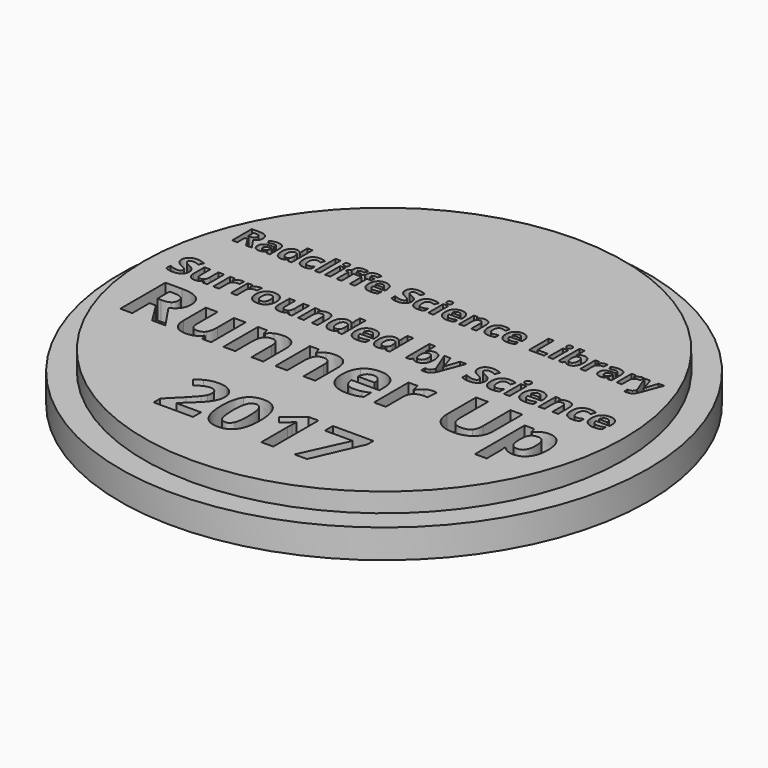
from build123d import *

# Parameters (mm, degrees)
F0_R           = 25
F0_W           = 0.5336082054
F0_H           = 1.9563767784
F0_H_2         = 2.7229136443
F0_W_2         = 0.6023027039
F0_H_3         = 2.2082325786
F1_DEPTH       = 5
F0_R_2         = 27.5
F0_TEXT_SIZE   = 8.2317518782
F0_TEXT_SIZE_2 = 4.0448450209
F0_TEXT_SIZE_3 = 3.583517854
F2_DEPTH       = 3


# Not quite as in the source:
# - Text() gives the source's letters only with a copy of the font that has no kerning and outlines rounded to 1/6400 em; it was checked with that copy


with BuildPart() as f1:
    # F0 (on Top) → F1 (new body)
    with BuildSketch(Plane.XY):
        Circle(F0_R)
        with BuildLine():
            Line((-4.7287555906, -17.9258199967), (-4.7287555906, -18.9715097275))
            Line((-4.7287555906, -18.9715097275), (-8.8369142623, -18.9715097275))
            Line((-8.8369142623, -18.9715097275), (-8.8369142623, -18.1071757803))
            Line((-8.8369142623, -18.1071757803), (-7.3616299804, -16.6164569636))
            add(Edge.make_bspline(
                [(-7.3616299804, -16.6164569636), (-6.7056622526, -15.9450547011), (-6.5050133006, -15.685883138)],
                knots=[0, 0, 0, 1, 1, 1], degree=2))
            add(Edge.make_bspline(
                [(-6.5050133006, -15.685883138), (-6.3043643486, -15.426711575), (-6.2156157736, -15.2054832433)],
                knots=[0, 0, 0, 1, 1, 1], degree=2))
            add(Edge.make_bspline(
                [(-6.2156157736, -15.2054832433), (-6.1268671987, -14.9842549115), (-6.1268671987, -14.747592045)],
                knots=[0, 0, 0, 1, 1, 1], degree=2))
            add(Edge.make_bspline(
                [(-6.1268671987, -14.747592045), (-6.1268671987, -14.3938839565), (-6.3223713058, -14.220888546)],
                knots=[0, 0, 0, 1, 1, 1], degree=2))
            add(Edge.make_bspline(
                [(-6.3223713058, -14.220888546), (-6.5178754129, -14.0478931354), (-6.8432868543, -14.0478931354)],
                knots=[0, 0, 0, 1, 1, 1], degree=2))
            add(Edge.make_bspline(
                [(-6.8432868543, -14.0478931354), (-7.1841328305, -14.0478931354), (-7.5056856383, -14.2048109056)],
                knots=[0, 0, 0, 1, 1, 1], degree=2))
            add(Edge.make_bspline(
                [(-7.5056856383, -14.2048109056), (-7.827238446, -14.3617286758), (-8.1770879008, -14.6511262027)],
                knots=[0, 0, 0, 1, 1, 1], degree=2))
            Line((-8.1770879008, -14.6511262027), (-8.8523487971, -13.8511028171))
            add(Edge.make_bspline(
                [(-8.8523487971, -13.8511028171), (-8.4188956123, -13.4806739825), (-8.133356719, -13.3282579517)],
                knots=[0, 0, 0, 1, 1, 1], degree=2))
            add(Edge.make_bspline(
                [(-8.133356719, -13.3282579517), (-7.8478178257, -13.1758419208), (-7.5101873776, -13.093524402)],
                knots=[0, 0, 0, 1, 1, 1], degree=2))
            add(Edge.make_bspline(
                [(-7.5101873776, -13.093524402), (-7.1725569295, -13.0112068832), (-6.7545382794, -13.0112068832)],
                knots=[0, 0, 0, 1, 1, 1], degree=2))
            add(Edge.make_bspline(
                [(-6.7545382794, -13.0112068832), (-6.2040398725, -13.0112068832), (-5.7821625888, -13.2118558353)],
                knots=[0, 0, 0, 1, 1, 1], degree=2))
            add(Edge.make_bspline(
                [(-5.7821625888, -13.2118558353), (-5.360285305, -13.4125047873), (-5.1268379666, -13.7745732488)],
                knots=[0, 0, 0, 1, 1, 1], degree=2))
            add(Edge.make_bspline(
                [(-5.1268379666, -13.7745732488), (-4.8933906282, -14.1366417103), (-4.8933906282, -14.6022501759)],
                knots=[0, 0, 0, 1, 1, 1], degree=2))
            add(Edge.make_bspline(
                [(-4.8933906282, -14.6022501759), (-4.8933906282, -15.0086929249), (-5.0361600748, -15.3643303303)],
                knots=[0, 0, 0, 1, 1, 1], degree=2))
            add(Edge.make_bspline(
                [(-5.0361600748, -15.3643303303), (-5.1789295215, -15.7199677356), (-5.4786167383, -16.0936120982)],
                knots=[0, 0, 0, 1, 1, 1], degree=2))
            add(Edge.make_bspline(
                [(-5.4786167383, -16.0936120982), (-5.7783039551, -16.4672564608), (-6.5333099477, -17.1592381031)],
                knots=[0, 0, 0, 1, 1, 1], degree=2))
            Line((-6.5333099477, -17.1592381031), (-7.2896021515, -17.8705129138))
            Line((-7.2896021515, -17.8705129138), (-7.2896021515, -17.9258199967))
            Line((-7.2896021515, -17.9258199967), (-4.7287555906, -17.9258199967))
        make_face(mode=Mode.SUBTRACT)
        with BuildLine():
            add(Edge.make_bspline(
                [(-0.5826536876, -13.7739301432), (-0.0623812447, -14.5456568818), (-0.0623812447, -16.033803276)],
                knots=[0, 0, 0, 1, 1, 1], degree=2))
            add(Edge.make_bspline(
                [(-0.0623812447, -16.033803276), (-0.0623812447, -17.5721119082), (-0.5665760472, -18.3123264717)],
                knots=[0, 0, 0, 1, 1, 1], degree=2))
            add(Edge.make_bspline(
                [(-0.5665760472, -18.3123264717), (-1.0707708498, -19.0525410351), (-2.1203192142, -19.0525410351)],
                knots=[0, 0, 0, 1, 1, 1], degree=2))
            add(Edge.make_bspline(
                [(-2.1203192142, -19.0525410351), (-3.1377122979, -19.0525410351), (-3.6541261072, -18.2885315639)],
                knots=[0, 0, 0, 1, 1, 1], degree=2))
            add(Edge.make_bspline(
                [(-3.6541261072, -18.2885315639), (-4.1705399164, -17.5245220927), (-4.1705399164, -16.033803276)],
                knots=[0, 0, 0, 1, 1, 1], degree=2))
            add(Edge.make_bspline(
                [(-4.1705399164, -16.033803276), (-4.1705399164, -14.4774876865), (-3.6676313251, -13.7398455456)],
                knots=[0, 0, 0, 1, 1, 1], degree=2))
            add(Edge.make_bspline(
                [(-3.6676313251, -13.7398455456), (-3.1647227338, -13.0022034046), (-2.1203192142, -13.0022034046)],
                knots=[0, 0, 0, 1, 1, 1], degree=2))
            add(Edge.make_bspline(
                [(-2.1203192142, -13.0022034046), (-1.1029261306, -13.0022034046), (-0.5826536876, -13.7739301432)],
                knots=[0, 0, 0, 1, 1, 1], degree=2))
        make_face(mode=Mode.SUBTRACT)
        with BuildLine():
            Line((-19.3516910754, -5.5215988853), (-20.0140898594, -5.5215988853))
            Line((-20.0140898594, -5.5215988853), (-20.0140898594, -7.7763271732))
            Line((-20.0140898594, -7.7763271732), (-21.2604285422, -7.7763271732))
            Line((-21.2604285422, -7.7763271732), (-21.2604285422, -1.899628059))
            Line((-21.2604285422, -1.899628059), (-19.5484813938, -1.899628059))
            add(Edge.make_bspline(
                [(-19.5484813938, -1.899628059), (-18.3497325265, -1.899628059), (-17.7754392119, -2.3356536662)],
                knots=[0, 0, 0, 1, 1, 1], degree=2))
            add(Edge.make_bspline(
                [(-17.7754392119, -2.3356536662), (-17.2011458973, -2.7716792735), (-17.2011458973, -3.6604512341)],
                knots=[0, 0, 0, 1, 1, 1], degree=2))
            add(Edge.make_bspline(
                [(-17.2011458973, -3.6604512341), (-17.2011458973, -4.1787943602), (-17.4860416849, -4.5826646867)],
                knots=[0, 0, 0, 1, 1, 1], degree=2))
            add(Edge.make_bspline(
                [(-17.4860416849, -4.5826646867), (-17.7709374726, -4.9865350133), (-18.2944254436, -5.2154806124)],
                knots=[0, 0, 0, 1, 1, 1], degree=2))
            add(Edge.make_bspline(
                [(-18.2944254436, -5.2154806124), (-16.9670554532, -7.1975321193), (-16.5657575492, -7.7763271732)],
                knots=[0, 0, 0, 1, 1, 1], degree=2))
            Line((-16.5657575492, -7.7763271732), (-17.9484346225, -7.7763271732))
            Line((-17.9484346225, -7.7763271732), (-19.3516910754, -5.5215988853))
        make_face(mode=Mode.SUBTRACT)
        with BuildLine():
            Line((-11.7990587272, -7.7763271732), (-12.7392791371, -7.7763271732))
            Line((-12.7392791371, -7.7763271732), (-12.9039141746, -7.201390753))
            Line((-12.9039141746, -7.201390753), (-12.9682247362, -7.201390753))
            add(Edge.make_bspline(
                [(-12.9682247362, -7.201390753), (-13.1650150545, -7.5152262933), (-13.527083516, -7.6862923871)],
                knots=[0, 0, 0, 1, 1, 1], degree=2))
            add(Edge.make_bspline(
                [(-13.527083516, -7.6862923871), (-13.8891519775, -7.8573584808), (-14.3509018095, -7.8573584808)],
                knots=[0, 0, 0, 1, 1, 1], degree=2))
            add(Edge.make_bspline(
                [(-14.3509018095, -7.8573584808), (-15.1432079277, -7.8573584808), (-15.5451489374, -7.4329087746)],
                knots=[0, 0, 0, 1, 1, 1], degree=2))
            add(Edge.make_bspline(
                [(-15.5451489374, -7.4329087746), (-15.9470899471, -7.0084590683), (-15.9470899471, -6.2122943164)],
                knots=[0, 0, 0, 1, 1, 1], degree=2))
            Line((-15.9470899471, -6.2122943164), (-15.9470899471, -3.2823051322))
            Line((-15.9470899471, -3.2823051322), (-14.721330644, -3.2823051322))
            Line((-14.721330644, -3.2823051322), (-14.721330644, -5.9074622546))
            add(Edge.make_bspline(
                [(-14.721330644, -5.9074622546), (-14.721330644, -6.3936500999), (-14.5483352334, -6.6367440226)],
                knots=[0, 0, 0, 1, 1, 1], degree=2))
            add(Edge.make_bspline(
                [(-14.5483352334, -6.6367440226), (-14.3753398229, -6.8798379452), (-13.997193721, -6.8798379452)],
                knots=[0, 0, 0, 1, 1, 1], degree=2))
            add(Edge.make_bspline(
                [(-13.997193721, -6.8798379452), (-13.4827092286, -6.8798379452), (-13.2537636295, -6.5364195466)],
                knots=[0, 0, 0, 1, 1, 1], degree=2))
            add(Edge.make_bspline(
                [(-13.2537636295, -6.5364195466), (-13.0248180303, -6.1930011479), (-13.0248180303, -5.3968363959)],
                knots=[0, 0, 0, 1, 1, 1], degree=2))
            Line((-13.0248180303, -5.3968363959), (-13.0248180303, -3.2823051322))
            Line((-13.0248180303, -3.2823051322), (-11.7990587272, -3.2823051322))
            Line((-11.7990587272, -3.2823051322), (-11.7990587272, -7.7763271732))
        make_face(mode=Mode.SUBTRACT)
        with BuildLine():
            Line((-6.3648162764, -4.8463379891), (-6.3648162764, -7.7763271732))
            Line((-6.3648162764, -7.7763271732), (-7.5905755795, -7.7763271732))
            Line((-7.5905755795, -7.7763271732), (-7.5905755795, -5.1511700508))
            add(Edge.make_bspline(
                [(-7.5905755795, -5.1511700508), (-7.5905755795, -4.6649822055), (-7.7635709901, -4.4218882829)],
                knots=[0, 0, 0, 1, 1, 1], degree=2))
            add(Edge.make_bspline(
                [(-7.7635709901, -4.4218882829), (-7.9365664007, -4.1787943602), (-8.3147125026, -4.1787943602)],
                knots=[0, 0, 0, 1, 1, 1], degree=2))
            add(Edge.make_bspline(
                [(-8.3147125026, -4.1787943602), (-8.8291969949, -4.1787943602), (-9.0581425941, -4.5222127589)],
                knots=[0, 0, 0, 1, 1, 1], degree=2))
            add(Edge.make_bspline(
                [(-9.0581425941, -4.5222127589), (-9.2870881932, -4.8656311576), (-9.2870881932, -5.6617959095)],
                knots=[0, 0, 0, 1, 1, 1], degree=2))
            Line((-9.2870881932, -5.6617959095), (-9.2870881932, -7.7763271732))
            Line((-9.2870881932, -7.7763271732), (-10.5128474963, -7.7763271732))
            Line((-10.5128474963, -7.7763271732), (-10.5128474963, -3.2823051322))
            Line((-10.5128474963, -3.2823051322), (-9.5764857201, -3.2823051322))
            Line((-9.5764857201, -3.2823051322), (-9.4118506826, -3.8572415525))
            Line((-9.4118506826, -3.8572415525), (-9.3436814873, -3.8572415525))
            add(Edge.make_bspline(
                [(-9.3436814873, -3.8572415525), (-9.1378876904, -3.531830111), (-8.7783916513, -3.3652657566)],
                knots=[0, 0, 0, 1, 1, 1], degree=2))
            add(Edge.make_bspline(
                [(-8.7783916513, -3.3652657566), (-8.4188956123, -3.1987014022), (-7.961004414, -3.1987014022)],
                knots=[0, 0, 0, 1, 1, 1], degree=2))
            add(Edge.make_bspline(
                [(-7.961004414, -3.1987014022), (-7.1764155632, -3.1987014022), (-6.7706159198, -3.6225080028)],
                knots=[0, 0, 0, 1, 1, 1], degree=2))
            add(Edge.make_bspline(
                [(-6.7706159198, -3.6225080028), (-6.3648162764, -4.0463146034), (-6.3648162764, -4.8463379891)],
                knots=[0, 0, 0, 1, 1, 1], degree=2))
        make_face(mode=Mode.SUBTRACT)
        with BuildLine():
            Line((-0.955011839, -4.8463379891), (-0.955011839, -7.7763271732))
            Line((-0.955011839, -7.7763271732), (-2.1807711421, -7.7763271732))
            Line((-2.1807711421, -7.7763271732), (-2.1807711421, -5.1511700508))
            add(Edge.make_bspline(
                [(-2.1807711421, -5.1511700508), (-2.1807711421, -4.6649822055), (-2.3537665527, -4.4218882829)],
                knots=[0, 0, 0, 1, 1, 1], degree=2))
            add(Edge.make_bspline(
                [(-2.3537665527, -4.4218882829), (-2.5267619632, -4.1787943602), (-2.9049080651, -4.1787943602)],
                knots=[0, 0, 0, 1, 1, 1], degree=2))
            add(Edge.make_bspline(
                [(-2.9049080651, -4.1787943602), (-3.4193925575, -4.1787943602), (-3.6483381566, -4.5222127589)],
                knots=[0, 0, 0, 1, 1, 1], degree=2))
            add(Edge.make_bspline(
                [(-3.6483381566, -4.5222127589), (-3.8772837557, -4.8656311576), (-3.8772837557, -5.6617959095)],
                knots=[0, 0, 0, 1, 1, 1], degree=2))
            Line((-3.8772837557, -5.6617959095), (-3.8772837557, -7.7763271732))
            Line((-3.8772837557, -7.7763271732), (-5.1030430588, -7.7763271732))
            Line((-5.1030430588, -7.7763271732), (-5.1030430588, -3.2823051322))
            Line((-5.1030430588, -3.2823051322), (-4.1666812827, -3.2823051322))
            Line((-4.1666812827, -3.2823051322), (-4.0020462451, -3.8572415525))
            Line((-4.0020462451, -3.8572415525), (-3.9338770499, -3.8572415525))
            add(Edge.make_bspline(
                [(-3.9338770499, -3.8572415525), (-3.7280832529, -3.531830111), (-3.3685872139, -3.3652657566)],
                knots=[0, 0, 0, 1, 1, 1], degree=2))
            add(Edge.make_bspline(
                [(-3.3685872139, -3.3652657566), (-3.0090911748, -3.1987014022), (-2.5511999766, -3.1987014022)],
                knots=[0, 0, 0, 1, 1, 1], degree=2))
            add(Edge.make_bspline(
                [(-2.5511999766, -3.1987014022), (-1.7666111257, -3.1987014022), (-1.3608114824, -3.6225080028)],
                knots=[0, 0, 0, 1, 1, 1], degree=2))
            add(Edge.make_bspline(
                [(-1.3608114824, -3.6225080028), (-0.955011839, -4.0463146034), (-0.955011839, -4.8463379891)],
                knots=[0, 0, 0, 1, 1, 1], degree=2))
        make_face(mode=Mode.SUBTRACT)
        with BuildLine():
            Line((3.6316174106, -13.0948106133), (3.6316174106, -18.9715097275))
            Line((3.6316174106, -18.9715097275), (2.3891373615, -18.9715097275))
            Line((2.3891373615, -18.9715097275), (2.3891373615, -15.5707672329))
            Line((2.3891373615, -15.5707672329), (2.4019994738, -15.0125515586))
            Line((2.4019994738, -15.0125515586), (2.4212926423, -14.4016012239))
            add(Edge.make_bspline(
                [(2.4212926423, -14.4016012239), (2.1126019469, -14.7102919193), (1.9916980911, -14.8067577617)],
                knots=[0, 0, 0, 1, 1, 1], degree=2))
            Line((1.9916980911, -14.8067577617), (1.3164371949, -15.3495389011))
            Line((1.3164371949, -15.3495389011), (0.7170627613, -14.6022501759))
            Line((0.7170627613, -14.6022501759), (2.6103656932, -13.0948106133))
            Line((2.6103656932, -13.0948106133), (3.6316174106, -13.0948106133))
        make_face(mode=Mode.SUBTRACT)
        Polygon((7.1442602824, -18.9715097275), (5.8413283054, -18.9715097275), (8.0484667777, -14.1482176114), (5.1506328744, -14.1482176114), (5.1506328744, -13.1025278806), (9.3668332895, -13.1025278806), (9.3668332895, -13.8832580978), align=None, mode=Mode.SUBTRACT)
        with BuildLine():
            add(Edge.make_bspline(
                [(3.232891929, -7.7788995957), (2.8676079394, -7.8573584808), (2.3402613347, -7.8573584808)],
                knots=[0, 0, 0, 1, 1, 1], degree=2))
            add(Edge.make_bspline(
                [(2.3402613347, -7.8573584808), (1.255985267, -7.8573584808), (0.6450349323, -7.2579840471)],
                knots=[0, 0, 0, 1, 1, 1], degree=2))
            add(Edge.make_bspline(
                [(0.6450349323, -7.2579840471), (0.0340845976, -6.6586096135), (0.0340845976, -5.5614714335)],
                knots=[0, 0, 0, 1, 1, 1], degree=2))
            add(Edge.make_bspline(
                [(0.0340845976, -5.5614714335), (0.0340845976, -4.4321779727), (0.598731328, -3.8154396875)],
                knots=[0, 0, 0, 1, 1, 1], degree=2))
            add(Edge.make_bspline(
                [(0.598731328, -3.8154396875), (1.1633780584, -3.1987014022), (2.1601917624, -3.1987014022)],
                knots=[0, 0, 0, 1, 1, 1], degree=2))
            add(Edge.make_bspline(
                [(2.1601917624, -3.1987014022), (3.1119880733, -3.1987014022), (3.6425502061, -3.7408394361)],
                knots=[0, 0, 0, 1, 1, 1], degree=2))
            add(Edge.make_bspline(
                [(3.6425502061, -3.7408394361), (4.1731123389, -4.2829774699), (4.1731123389, -5.2399186258)],
                knots=[0, 0, 0, 1, 1, 1], degree=2))
            Line((4.1731123389, -5.2399186258), (4.1731123389, -5.8354344257))
            Line((4.1731123389, -5.8354344257), (1.2752784355, -5.8354344257))
            add(Edge.make_bspline(
                [(1.2752784355, -5.8354344257), (1.2958578152, -6.3576361855), (1.5852553422, -6.6508923461)],
                knots=[0, 0, 0, 1, 1, 1], degree=2))
            add(Edge.make_bspline(
                [(1.5852553422, -6.6508923461), (1.8746528691, -6.9441485068), (2.3968546289, -6.9441485068)],
                knots=[0, 0, 0, 1, 1, 1], degree=2))
            add(Edge.make_bspline(
                [(2.3968546289, -6.9441485068), (2.8032973779, -6.9441485068), (3.1647227338, -6.8599016712)],
                knots=[0, 0, 0, 1, 1, 1], degree=2))
            add(Edge.make_bspline(
                [(3.1647227338, -6.8599016712), (3.5261480897, -6.7756548355), (3.9197287264, -6.5904404183)],
                knots=[0, 0, 0, 1, 1, 1], degree=2))
            Line((3.9197287264, -6.5904404183), (3.9197287264, -7.5396643067))
            add(Edge.make_bspline(
                [(3.9197287264, -7.5396643067), (3.5981759186, -7.7004407106), (3.232891929, -7.7788995957)],
                knots=[0, 0, 0, 1, 1, 1], degree=2))
        make_face(mode=Mode.SUBTRACT)
        with BuildLine():
            add(Edge.make_bspline(
                [(6.9043818878, -3.4295763182), (7.2600192932, -3.1987014022), (7.6780379432, -3.1987014022)],
                knots=[0, 0, 0, 1, 1, 1], degree=2))
            add(Edge.make_bspline(
                [(7.6780379432, -3.1987014022), (7.927562922, -3.1987014022), (8.0921979596, -3.2347153167)],
                knots=[0, 0, 0, 1, 1, 1], degree=2))
            Line((8.0921979596, -3.2347153167), (7.999590751, -4.3833019459))
            add(Edge.make_bspline(
                [(7.999590751, -4.3833019459), (7.8503902482, -4.3434293978), (7.6381653951, -4.3434293978)],
                knots=[0, 0, 0, 1, 1, 1], degree=2))
            add(Edge.make_bspline(
                [(7.6381653951, -4.3434293978), (7.0516530738, -4.3434293978), (6.7236692099, -4.6450459314)],
                knots=[0, 0, 0, 1, 1, 1], degree=2))
            add(Edge.make_bspline(
                [(6.7236692099, -4.6450459314), (6.395685346, -4.9466624651), (6.395685346, -5.4894436046)],
                knots=[0, 0, 0, 1, 1, 1], degree=2))
            Line((6.395685346, -5.4894436046), (6.395685346, -7.7763271732))
            Line((6.395685346, -7.7763271732), (5.1699260429, -7.7763271732))
            Line((5.1699260429, -7.7763271732), (5.1699260429, -3.2823051322))
            Line((5.1699260429, -3.2823051322), (6.0985705516, -3.2823051322))
            Line((6.0985705516, -3.2823051322), (6.2799263352, -4.038597336))
            Line((6.2799263352, -4.038597336), (6.3390920518, -4.038597336))
            add(Edge.make_bspline(
                [(6.3390920518, -4.038597336), (6.5487444824, -3.6604512341), (6.9043818878, -3.4295763182)],
                knots=[0, 0, 0, 1, 1, 1], degree=2))
        make_face(mode=Mode.SUBTRACT)
        with BuildLine():
            Line((14.6840305183, -1.899628059), (15.9265105674, -1.899628059))
            Line((15.9265105674, -1.899628059), (15.9265105674, -5.7016684577))
            add(Edge.make_bspline(
                [(15.9265105674, -5.7016684577), (15.9265105674, -6.3537775518), (15.6351837236, -6.8438240308)],
                knots=[0, 0, 0, 1, 1, 1], degree=2))
            add(Edge.make_bspline(
                [(15.6351837236, -6.8438240308), (15.3438568798, -7.3338705098), (14.7927153673, -7.5956144953)],
                knots=[0, 0, 0, 1, 1, 1], degree=2))
            add(Edge.make_bspline(
                [(14.7927153673, -7.5956144953), (14.2415738548, -7.8573584808), (13.490426496, -7.8573584808)],
                knots=[0, 0, 0, 1, 1, 1], degree=2))
            add(Edge.make_bspline(
                [(13.490426496, -7.8573584808), (12.3572744015, -7.8573584808), (11.7302464264, -7.2759910044)],
                knots=[0, 0, 0, 1, 1, 1], degree=2))
            add(Edge.make_bspline(
                [(11.7302464264, -7.2759910044), (11.1032184513, -6.694623528), (11.1032184513, -5.6862339229)],
                knots=[0, 0, 0, 1, 1, 1], degree=2))
            Line((11.1032184513, -5.6862339229), (11.1032184513, -1.899628059))
            Line((11.1032184513, -1.899628059), (12.3444122892, -1.899628059))
            Line((12.3444122892, -1.899628059), (12.3444122892, -5.497160872))
            add(Edge.make_bspline(
                [(12.3444122892, -5.497160872), (12.3444122892, -6.1762804019), (12.6177321757, -6.493974576)],
                knots=[0, 0, 0, 1, 1, 1], degree=2))
            add(Edge.make_bspline(
                [(12.6177321757, -6.493974576), (12.8910520623, -6.81166875), (13.5225817767, -6.81166875)],
                knots=[0, 0, 0, 1, 1, 1], degree=2))
            add(Edge.make_bspline(
                [(13.5225817767, -6.81166875), (14.1335321114, -6.81166875), (14.4087813149, -6.4920452591)],
                knots=[0, 0, 0, 1, 1, 1], degree=2))
            add(Edge.make_bspline(
                [(14.4087813149, -6.4920452591), (14.6840305183, -6.1724217682), (14.6840305183, -5.4894436046)],
                knots=[0, 0, 0, 1, 1, 1], degree=2))
            Line((14.6840305183, -5.4894436046), (14.6840305183, -1.899628059))
        make_face(mode=Mode.SUBTRACT)
        with BuildLine():
            add(Edge.make_bspline(
                [(20.6533368412, -7.5795368549), (20.2636148382, -7.8573584808), (19.7375544447, -7.8573584808)],
                knots=[0, 0, 0, 1, 1, 1], degree=2))
            add(Edge.make_bspline(
                [(19.7375544447, -7.8573584808), (18.9452483265, -7.8573584808), (18.4950743956, -7.2824220605)],
                knots=[0, 0, 0, 1, 1, 1], degree=2))
            Line((18.4950743956, -7.2824220605), (18.4307638341, -7.2824220605))
            add(Edge.make_bspline(
                [(18.4307638341, -7.2824220605), (18.4950743956, -7.8444963685), (18.4950743956, -7.9332449434)],
                knots=[0, 0, 0, 1, 1, 1], degree=2))
            Line((18.4950743956, -7.9332449434), (18.4950743956, -9.7545200464))
            Line((18.4950743956, -9.7545200464), (17.2693150925, -9.7545200464))
            Line((17.2693150925, -9.7545200464), (17.2693150925, -3.2823051322))
            Line((17.2693150925, -3.2823051322), (18.2661287965, -3.2823051322))
            Line((18.2661287965, -3.2823051322), (18.4384811015, -3.8649588199))
            Line((18.4384811015, -3.8649588199), (18.4950743956, -3.8649588199))
            add(Edge.make_bspline(
                [(18.4950743956, -3.8649588199), (18.925955158, -3.1987014022), (19.7697097255, -3.1987014022)],
                knots=[0, 0, 0, 1, 1, 1], degree=2))
            add(Edge.make_bspline(
                [(19.7697097255, -3.1987014022), (20.5658744775, -3.1987014022), (21.0160484083, -3.8135103706)],
                knots=[0, 0, 0, 1, 1, 1], degree=2))
            add(Edge.make_bspline(
                [(21.0160484083, -3.8135103706), (21.4662223392, -4.428319339), (21.4662223392, -5.5215988853)],
                knots=[0, 0, 0, 1, 1, 1], degree=2))
            add(Edge.make_bspline(
                [(21.4662223392, -5.5215988853), (21.4662223392, -6.2405909635), (21.2546405917, -6.7711530962)],
                knots=[0, 0, 0, 1, 1, 1], degree=2))
            add(Edge.make_bspline(
                [(21.2546405917, -6.7711530962), (21.0430588442, -7.301715229), (20.6533368412, -7.5795368549)],
                knots=[0, 0, 0, 1, 1, 1], degree=2))
        make_face(mode=Mode.SUBTRACT)
        with BuildLine():
            add(Edge.make_bspline(
                [(-21.0821746538, 1.2788662343), (-20.9320729831, 1.0845240712), (-20.9320729831, 0.8020169268)],
                knots=[0, 0, 0, 1, 1, 1], degree=2))
            add(Edge.make_bspline(
                [(-20.9320729831, 0.8020169268), (-20.9320729831, 0.4108045724), (-21.2136321169, 0.1854940646)],
                knots=[0, 0, 0, 1, 1, 1], degree=2))
            add(Edge.make_bspline(
                [(-21.2136321169, 0.1854940646), (-21.4951912508, -0.0398164432), (-21.9963728292, -0.0398164432)],
                knots=[0, 0, 0, 1, 1, 1], degree=2))
            add(Edge.make_bspline(
                [(-21.9963728292, -0.0398164432), (-22.4590019785, -0.0398164432), (-22.8141899319, 0.1346174984)],
                knots=[0, 0, 0, 1, 1, 1], degree=2))
            Line((-22.8141899319, 0.1346174984), (-22.8141899319, 0.7034238294))
            add(Edge.make_bspline(
                [(-22.8141899319, 0.7034238294), (-22.5222026819, 0.5725983733), (-22.3196444273, 0.5195097824)],
                knots=[0, 0, 0, 1, 1, 1], degree=2))
            add(Edge.make_bspline(
                [(-22.3196444273, 0.5195097824), (-22.1170861728, 0.4664211915), (-21.9489723016, 0.4664211915)],
                knots=[0, 0, 0, 1, 1, 1], degree=2))
            add(Edge.make_bspline(
                [(-21.9489723016, 0.4664211915), (-21.7479940646, 0.4664211915), (-21.6402368652, 0.5432100462)],
                knots=[0, 0, 0, 1, 1, 1], degree=2))
            add(Edge.make_bspline(
                [(-21.6402368652, 0.5432100462), (-21.5324796659, 0.6199989009), (-21.5324796659, 0.7723125962)],
                knots=[0, 0, 0, 1, 1, 1], degree=2))
            add(Edge.make_bspline(
                [(-21.5324796659, 0.7723125962), (-21.5324796659, 0.8570015388), (-21.5798801934, 0.9233622774)],
                knots=[0, 0, 0, 1, 1, 1], degree=2))
            add(Edge.make_bspline(
                [(-21.5798801934, 0.9233622774), (-21.627280721, 0.989723016), (-21.7192377446, 1.0507116949)],
                knots=[0, 0, 0, 1, 1, 1], degree=2))
            add(Edge.make_bspline(
                [(-21.7192377446, 1.0507116949), (-21.8111947681, 1.1117003737), (-22.0937019125, 1.2463178721)],
                knots=[0, 0, 0, 1, 1, 1], degree=2))
            add(Edge.make_bspline(
                [(-22.0937019125, 1.2463178721), (-22.3578808529, 1.3708232579), (-22.4902863267, 1.4852165311)],
                knots=[0, 0, 0, 1, 1, 1], degree=2))
            add(Edge.make_bspline(
                [(-22.4902863267, 1.4852165311), (-22.6226918004, 1.5996098044), (-22.7016926797, 1.7519234997)],
                knots=[0, 0, 0, 1, 1, 1], degree=2))
            add(Edge.make_bspline(
                [(-22.7016926797, 1.7519234997), (-22.780693559, 1.904237195), (-22.780693559, 2.1071114531)],
                knots=[0, 0, 0, 1, 1, 1], degree=2))
            add(Edge.make_bspline(
                [(-22.780693559, 2.1071114531), (-22.780693559, 2.490739723), (-22.5209386678, 2.7097301605)],
                knots=[0, 0, 0, 1, 1, 1], degree=2))
            add(Edge.make_bspline(
                [(-22.5209386678, 2.7097301605), (-22.2611837767, 2.9287205979), (-21.8029786766, 2.9287205979)],
                knots=[0, 0, 0, 1, 1, 1], degree=2))
            add(Edge.make_bspline(
                [(-21.8029786766, 2.9287205979), (-21.5779841723, 2.9287205979), (-21.3735298967, 2.875632007)],
                knots=[0, 0, 0, 1, 1, 1], degree=2))
            add(Edge.make_bspline(
                [(-21.3735298967, 2.875632007), (-21.169075621, 2.8225434161), (-20.9459771378, 2.7258463399)],
                knots=[0, 0, 0, 1, 1, 1], degree=2))
            Line((-20.9459771378, 2.7258463399), (-21.1431633326, 2.2493130358))
            add(Edge.make_bspline(
                [(-21.1431633326, 2.2493130358), (-21.3744779072, 2.344114091), (-21.5255275885, 2.3817185096)],
                knots=[0, 0, 0, 1, 1, 1], degree=2))
            add(Edge.make_bspline(
                [(-21.5255275885, 2.3817185096), (-21.6765772697, 2.4193229281), (-21.8225708947, 2.4193229281)],
                knots=[0, 0, 0, 1, 1, 1], degree=2))
            add(Edge.make_bspline(
                [(-21.8225708947, 2.4193229281), (-21.9963728292, 2.4193229281), (-22.0892778633, 2.3384260277)],
                knots=[0, 0, 0, 1, 1, 1], degree=2))
            add(Edge.make_bspline(
                [(-22.0892778633, 2.3384260277), (-22.1821828973, 2.2575291273), (-22.1821828973, 2.1273356782)],
                knots=[0, 0, 0, 1, 1, 1], degree=2))
            add(Edge.make_bspline(
                [(-22.1821828973, 2.1273356782), (-22.1821828973, 2.0464387778), (-22.1445784788, 1.986082106)],
                knots=[0, 0, 0, 1, 1, 1], degree=2))
            add(Edge.make_bspline(
                [(-22.1445784788, 1.986082106), (-22.1069740602, 1.9257254342), (-22.0251291493, 1.8694768081)],
                knots=[0, 0, 0, 1, 1, 1], degree=2))
            add(Edge.make_bspline(
                [(-22.0251291493, 1.8694768081), (-21.9432842383, 1.813228182), (-21.6373928336, 1.667234557)],
                knots=[0, 0, 0, 1, 1, 1], degree=2))
            add(Edge.make_bspline(
                [(-21.6373928336, 1.667234557), (-21.2322763245, 1.4732083974), (-21.0821746538, 1.2788662343)],
                knots=[0, 0, 0, 1, 1, 1], degree=2))
        make_face(mode=Mode.SUBTRACT)
        with BuildLine():
            Line((-18.4299571334, 0), (-18.8919542757, 0))
            Line((-18.8919542757, 0), (-18.9728511761, 0.2825071444))
            Line((-18.9728511761, 0.2825071444), (-19.0044515278, 0.2825071444))
            add(Edge.make_bspline(
                [(-19.0044515278, 0.2825071444), (-19.1011486041, 0.128297428), (-19.2790585843, 0.0442404924)],
                knots=[0, 0, 0, 1, 1, 1], degree=2))
            add(Edge.make_bspline(
                [(-19.2790585843, 0.0442404924), (-19.4569685645, -0.0398164432), (-19.6838590899, -0.0398164432)],
                knots=[0, 0, 0, 1, 1, 1], degree=2))
            add(Edge.make_bspline(
                [(-19.6838590899, -0.0398164432), (-20.0731754232, -0.0398164432), (-20.2706776215, 0.1687458782)],
                knots=[0, 0, 0, 1, 1, 1], degree=2))
            add(Edge.make_bspline(
                [(-20.2706776215, 0.1687458782), (-20.4681798197, 0.3773081996), (-20.4681798197, 0.768520554)],
                knots=[0, 0, 0, 1, 1, 1], degree=2))
            Line((-20.4681798197, 0.768520554), (-20.4681798197, 2.2082325786))
            Line((-20.4681798197, 2.2082325786), (-19.8658771158, 2.2082325786))
            Line((-19.8658771158, 2.2082325786), (-19.8658771158, 0.9183062211))
            add(Edge.make_bspline(
                [(-19.8658771158, 0.9183062211), (-19.8658771158, 0.6794075621), (-19.7808721697, 0.5599582326)],
                knots=[0, 0, 0, 1, 1, 1], degree=2))
            add(Edge.make_bspline(
                [(-19.7808721697, 0.5599582326), (-19.6958672236, 0.4405089031), (-19.5100571554, 0.4405089031)],
                knots=[0, 0, 0, 1, 1, 1], degree=2))
            add(Edge.make_bspline(
                [(-19.5100571554, 0.4405089031), (-19.2572543416, 0.4405089031), (-19.1447570895, 0.6092547813)],
                knots=[0, 0, 0, 1, 1, 1], degree=2))
            add(Edge.make_bspline(
                [(-19.1447570895, 0.6092547813), (-19.0322598373, 0.7780006595), (-19.0322598373, 1.1692130138)],
                knots=[0, 0, 0, 1, 1, 1], degree=2))
            Line((-19.0322598373, 1.1692130138), (-19.0322598373, 2.2082325786))
            Line((-19.0322598373, 2.2082325786), (-18.4299571334, 2.2082325786))
            Line((-18.4299571334, 2.2082325786), (-18.4299571334, 0))
        make_face(mode=Mode.SUBTRACT)
        with BuildLine():
            add(Edge.make_bspline(
                [(-16.9456886129, 2.1358677731), (-16.7709386678, 2.2493130358), (-16.5655363816, 2.2493130358)],
                knots=[0, 0, 0, 1, 1, 1], degree=2))
            add(Edge.make_bspline(
                [(-16.5655363816, 2.2493130358), (-16.4429270169, 2.2493130358), (-16.3620301165, 2.2316168389)],
                knots=[0, 0, 0, 1, 1, 1], degree=2))
            Line((-16.3620301165, 2.2316168389), (-16.407534623, 1.667234557))
            add(Edge.make_bspline(
                [(-16.407534623, 1.667234557), (-16.480847439, 1.6868267751), (-16.5851285997, 1.6868267751)],
                knots=[0, 0, 0, 1, 1, 1], degree=2))
            add(Edge.make_bspline(
                [(-16.5851285997, 1.6868267751), (-16.8733238074, 1.6868267751), (-17.0344856012, 1.5386211255)],
                knots=[0, 0, 0, 1, 1, 1], degree=2))
            add(Edge.make_bspline(
                [(-17.0344856012, 1.5386211255), (-17.195647395, 1.3904154759), (-17.195647395, 1.1237085074)],
                knots=[0, 0, 0, 1, 1, 1], degree=2))
            Line((-17.195647395, 1.1237085074), (-17.195647395, 0))
            Line((-17.195647395, 0), (-17.7979500989, 0))
            Line((-17.7979500989, 0), (-17.7979500989, 2.2082325786))
            Line((-17.7979500989, 2.2082325786), (-17.34164102, 2.2082325786))
            Line((-17.34164102, 2.2082325786), (-17.2525280281, 1.8366124423))
            Line((-17.2525280281, 1.8366124423), (-17.2234557046, 1.8366124423))
            add(Edge.make_bspline(
                [(-17.2234557046, 1.8366124423), (-17.1204385579, 2.0224225104), (-16.9456886129, 2.1358677731)],
                knots=[0, 0, 0, 1, 1, 1], degree=2))
        make_face(mode=Mode.SUBTRACT)
        with BuildLine():
            add(Edge.make_bspline(
                [(-15.1090761706, 2.1358677731), (-14.9343262255, 2.2493130358), (-14.7289239393, 2.2493130358)],
                knots=[0, 0, 0, 1, 1, 1], degree=2))
            add(Edge.make_bspline(
                [(-14.7289239393, 2.2493130358), (-14.6063145746, 2.2493130358), (-14.5254176742, 2.2316168389)],
                knots=[0, 0, 0, 1, 1, 1], degree=2))
            Line((-14.5254176742, 2.2316168389), (-14.5709221807, 1.667234557))
            add(Edge.make_bspline(
                [(-14.5709221807, 1.667234557), (-14.6442349967, 1.6868267751), (-14.7485161574, 1.6868267751)],
                knots=[0, 0, 0, 1, 1, 1], degree=2))
            add(Edge.make_bspline(
                [(-14.7485161574, 1.6868267751), (-15.0367113651, 1.6868267751), (-15.1978731589, 1.5386211255)],
                knots=[0, 0, 0, 1, 1, 1], degree=2))
            add(Edge.make_bspline(
                [(-15.1978731589, 1.5386211255), (-15.3590349527, 1.3904154759), (-15.3590349527, 1.1237085074)],
                knots=[0, 0, 0, 1, 1, 1], degree=2))
            Line((-15.3590349527, 1.1237085074), (-15.3590349527, 0))
            Line((-15.3590349527, 0), (-15.9613376566, 0))
            Line((-15.9613376566, 0), (-15.9613376566, 2.2082325786))
            Line((-15.9613376566, 2.2082325786), (-15.5050285777, 2.2082325786))
            Line((-15.5050285777, 2.2082325786), (-15.4159155858, 1.8366124423))
            Line((-15.4159155858, 1.8366124423), (-15.3868432623, 1.8366124423))
            add(Edge.make_bspline(
                [(-15.3868432623, 1.8366124423), (-15.2838261156, 2.0224225104), (-15.1090761706, 2.1358677731)],
                knots=[0, 0, 0, 1, 1, 1], degree=2))
        make_face(mode=Mode.SUBTRACT)
        with BuildLine():
            Line((-20.8471151154, 8.2907262753), (-21.1354763177, 8.2907262753))
            Line((-21.1354763177, 8.2907262753), (-21.1354763177, 7.3091783382))
            Line((-21.1354763177, 7.3091783382), (-21.6780433178, 7.3091783382))
            Line((-21.6780433178, 7.3091783382), (-21.6780433178, 9.8674741311))
            Line((-21.6780433178, 9.8674741311), (-20.9327835891, 9.8674741311))
            add(Edge.make_bspline(
                [(-20.9327835891, 9.8674741311), (-20.4109338016, 9.8674741311), (-20.1609274389, 9.6776596698)],
                knots=[0, 0, 0, 1, 1, 1], degree=2))
            add(Edge.make_bspline(
                [(-20.1609274389, 9.6776596698), (-19.9109210761, 9.4878452084), (-19.9109210761, 9.1009372651)],
                knots=[0, 0, 0, 1, 1, 1], degree=2))
            add(Edge.make_bspline(
                [(-19.9109210761, 9.1009372651), (-19.9109210761, 8.8752876253), (-20.0349443893, 8.6994712806)],
                knots=[0, 0, 0, 1, 1, 1], degree=2))
            add(Edge.make_bspline(
                [(-20.0349443893, 8.6994712806), (-20.1589677025, 8.5236549359), (-20.3868570411, 8.4239883455)],
                knots=[0, 0, 0, 1, 1, 1], degree=2))
            add(Edge.make_bspline(
                [(-20.3868570411, 8.4239883455), (-19.8090147871, 7.5611444373), (-19.6343182917, 7.3091783382)],
                knots=[0, 0, 0, 1, 1, 1], degree=2))
            Line((-19.6343182917, 7.3091783382), (-20.2362373063, 7.3091783382))
            Line((-20.2362373063, 7.3091783382), (-20.8471151154, 8.2907262753))
        make_face(mode=Mode.SUBTRACT)
        with BuildLine():
            Line((-17.7395332264, 7.3091783382), (-18.1118831285, 7.3091783382))
            Line((-18.1118831285, 7.3091783382), (-18.2154691914, 7.5751425539))
            Line((-18.2154691914, 7.5751425539), (-18.229467308, 7.5751425539))
            add(Edge.make_bspline(
                [(-18.229467308, 7.5751425539), (-18.3638492276, 7.4054853805), (-18.5066300171, 7.3396942324)],
                knots=[0, 0, 0, 1, 1, 1], degree=2))
            add(Edge.make_bspline(
                [(-18.5066300171, 7.3396942324), (-18.6494108065, 7.2739030843), (-18.8784199944, 7.2739030843)],
                knots=[0, 0, 0, 1, 1, 1], degree=2))
            add(Edge.make_bspline(
                [(-18.8784199944, 7.2739030843), (-19.1600621007, 7.2739030843), (-19.3218803288, 7.4351613877)],
                knots=[0, 0, 0, 1, 1, 1], degree=2))
            add(Edge.make_bspline(
                [(-19.3218803288, 7.4351613877), (-19.4836985569, 7.5964196911), (-19.4836985569, 7.8937396881)],
                knots=[0, 0, 0, 1, 1, 1], degree=2))
            add(Edge.make_bspline(
                [(-19.4836985569, 7.8937396881), (-19.4836985569, 8.2050578016), (-19.2658878624, 8.3528779131)],
                knots=[0, 0, 0, 1, 1, 1], degree=2))
            add(Edge.make_bspline(
                [(-19.2658878624, 8.3528779131), (-19.0480771678, 8.5006980246), (-18.6090962307, 8.5163759152)],
                knots=[0, 0, 0, 1, 1, 1], degree=2))
            Line((-18.6090962307, 8.5163759152), (-18.2692219592, 8.5270144838))
            Line((-18.2692219592, 8.5270144838), (-18.2692219592, 8.6126829575))
            add(Edge.make_bspline(
                [(-18.2692219592, 8.6126829575), (-18.2692219592, 8.9100029545), (-18.5738209768, 8.9100029545)],
                knots=[0, 0, 0, 1, 1, 1], degree=2))
            add(Edge.make_bspline(
                [(-18.5738209768, 8.9100029545), (-18.8084294113, 8.9100029545), (-19.1253467715, 8.7683420143)],
                knots=[0, 0, 0, 1, 1, 1], degree=2))
            Line((-19.1253467715, 8.7683420143), (-19.3017230409, 9.1289334984))
            add(Edge.make_bspline(
                [(-19.3017230409, 9.1289334984), (-18.9640884681, 9.3058696924), (-18.5531037642, 9.3058696924)],
                knots=[0, 0, 0, 1, 1, 1], degree=2))
            add(Edge.make_bspline(
                [(-18.5531037642, 9.3058696924), (-18.1594767249, 9.3058696924), (-17.9495049757, 9.1342527827)],
                knots=[0, 0, 0, 1, 1, 1], degree=2))
            add(Edge.make_bspline(
                [(-17.9495049757, 9.1342527827), (-17.7395332264, 8.962635873), (-17.7395332264, 8.6126829575)],
                knots=[0, 0, 0, 1, 1, 1], degree=2))
            Line((-17.7395332264, 8.6126829575), (-17.7395332264, 7.3091783382))
        make_face(mode=Mode.SUBTRACT)
        with BuildLine():
            add(Edge.make_bspline(
                [(-13.7943040391, 7.3055388278), (-13.92644626, 7.2739030843), (-14.1274592146, 7.2739030843)],
                knots=[0, 0, 0, 1, 1, 1], degree=2))
            add(Edge.make_bspline(
                [(-14.1274592146, 7.2739030843), (-15.0406963427, 7.2739030843), (-15.0406963427, 8.2767281587)],
                knots=[0, 0, 0, 1, 1, 1], degree=2))
            add(Edge.make_bspline(
                [(-15.0406963427, 8.2767281587), (-15.0406963427, 8.775621035), (-14.7923697539, 9.0387856274)],
                knots=[0, 0, 0, 1, 1, 1], degree=2))
            add(Edge.make_bspline(
                [(-14.7923697539, 9.0387856274), (-14.5440431651, 9.3019502198), (-14.0804255427, 9.3019502198)],
                knots=[0, 0, 0, 1, 1, 1], degree=2))
            add(Edge.make_bspline(
                [(-14.0804255427, 9.3019502198), (-13.7411111959, 9.3019502198), (-13.4712275076, 9.1692480742)],
                knots=[0, 0, 0, 1, 1, 1], degree=2))
            Line((-13.4712275076, 9.1692480742), (-13.629126263, 8.7560236717))
            add(Edge.make_bspline(
                [(-13.629126263, 8.7560236717), (-13.7551093126, 8.8069768162), (-13.8634547352, 8.8394524467)],
                knots=[0, 0, 0, 1, 1, 1], degree=2))
            add(Edge.make_bspline(
                [(-13.8634547352, 8.8394524467), (-13.9718001578, 8.8719280773), (-14.0804255427, 8.8719280773)],
                knots=[0, 0, 0, 1, 1, 1], degree=2))
            add(Edge.make_bspline(
                [(-14.0804255427, 8.8719280773), (-14.4970094933, 8.8719280773), (-14.4970094933, 8.2800877067)],
                knots=[0, 0, 0, 1, 1, 1], degree=2))
            add(Edge.make_bspline(
                [(-14.4970094933, 8.2800877067), (-14.4970094933, 7.7061649254), (-14.0804255427, 7.7061649254)],
                knots=[0, 0, 0, 1, 1, 1], degree=2))
            add(Edge.make_bspline(
                [(-14.0804255427, 7.7061649254), (-13.92644626, 7.7061649254), (-13.7951439261, 7.7473193883)],
                knots=[0, 0, 0, 1, 1, 1], degree=2))
            add(Edge.make_bspline(
                [(-13.7951439261, 7.7473193883), (-13.6638415922, 7.7884738511), (-13.5328192207, 7.8763820235)],
                knots=[0, 0, 0, 1, 1, 1], degree=2))
            Line((-13.5328192207, 7.8763820235), (-13.5328192207, 7.4194834971))
            add(Edge.make_bspline(
                [(-13.5328192207, 7.4194834971), (-13.6621618182, 7.3371745714), (-13.7943040391, 7.3055388278)],
                knots=[0, 0, 0, 1, 1, 1], degree=2))
        make_face(mode=Mode.SUBTRACT)
        with BuildLine():
            add(Edge.make_bspline(
                [(-16.0155251839, 7.5628242113), (-16.1975006999, 7.2739030843), (-16.5704105266, 7.2739030843)],
                knots=[0, 0, 0, 1, 1, 1], degree=2))
            add(Edge.make_bspline(
                [(-16.5704105266, 7.2739030843), (-16.9147641954, 7.2739030843), (-17.111577715, 7.5418270363)],
                knots=[0, 0, 0, 1, 1, 1], degree=2))
            add(Edge.make_bspline(
                [(-17.111577715, 7.5418270363), (-17.3083912346, 7.8097509884), (-17.3083912346, 8.2840071794)],
                knots=[0, 0, 0, 1, 1, 1], degree=2))
            add(Edge.make_bspline(
                [(-17.3083912346, 8.2840071794), (-17.3083912346, 8.7649824663), (-17.108218167, 9.033466343)],
                knots=[0, 0, 0, 1, 1, 1], degree=2))
            add(Edge.make_bspline(
                [(-17.108218167, 9.033466343), (-16.9080450994, 9.3019502198), (-16.55641241, 9.3019502198)],
                knots=[0, 0, 0, 1, 1, 1], degree=2))
            add(Edge.make_bspline(
                [(-16.55641241, 9.3019502198), (-16.1868621313, 9.3019502198), (-15.9925682726, 9.0152687914)],
                knots=[0, 0, 0, 1, 1, 1], degree=2))
            Line((-15.9925682726, 9.0152687914), (-15.975210608, 9.0152687914))
            add(Edge.make_bspline(
                [(-15.975210608, 9.0152687914), (-16.0155251839, 9.2341993353), (-16.0155251839, 9.4055362827)],
                knots=[0, 0, 0, 1, 1, 1], degree=2))
            Line((-16.0155251839, 9.4055362827), (-16.0155251839, 10.0320919825))
            Line((-16.0155251839, 10.0320919825), (-15.4802372044, 10.0320919825))
            Line((-15.4802372044, 10.0320919825), (-15.4802372044, 7.3091783382))
            Line((-15.4802372044, 7.3091783382), (-15.8895421343, 7.3091783382))
            Line((-15.8895421343, 7.3091783382), (-15.9925682726, 7.5628242113))
            Line((-15.9925682726, 7.5628242113), (-16.0155251839, 7.5628242113))
        make_face(mode=Mode.SUBTRACT)
        with BuildLine():
            add(Edge.make_bspline(
                [(-12.2482963289, 1.7143190811), (-12.1181028798, 1.4555122005), (-12.1181028798, 1.1079083315)],
                knots=[0, 0, 0, 1, 1, 1], degree=2))
            add(Edge.make_bspline(
                [(-12.1181028798, 1.1079083315), (-12.1181028798, 0.5688063311), (-12.4025060453, 0.2644949439)],
                knots=[0, 0, 0, 1, 1, 1], degree=2))
            add(Edge.make_bspline(
                [(-12.4025060453, 0.2644949439), (-12.6869092108, -0.0398164432), (-13.1944108595, -0.0398164432)],
                knots=[0, 0, 0, 1, 1, 1], degree=2))
            add(Edge.make_bspline(
                [(-13.1944108595, -0.0398164432), (-13.5123103979, -0.0398164432), (-13.7553171027, 0.0995411079)],
                knots=[0, 0, 0, 1, 1, 1], degree=2))
            add(Edge.make_bspline(
                [(-13.7553171027, 0.0995411079), (-13.9983238074, 0.238898659), (-14.1285172565, 0.4996015608)],
                knots=[0, 0, 0, 1, 1, 1], degree=2))
            add(Edge.make_bspline(
                [(-14.1285172565, 0.4996015608), (-14.2587107056, 0.7603044625), (-14.2587107056, 1.1079083315)],
                knots=[0, 0, 0, 1, 1, 1], degree=2))
            add(Edge.make_bspline(
                [(-14.2587107056, 1.1079083315), (-14.2587107056, 1.648906353), (-13.9765195647, 1.9491096944)],
                knots=[0, 0, 0, 1, 1, 1], degree=2))
            add(Edge.make_bspline(
                [(-13.9765195647, 1.9491096944), (-13.6943284238, 2.2493130358), (-13.1824027259, 2.2493130358)],
                knots=[0, 0, 0, 1, 1, 1], degree=2))
            add(Edge.make_bspline(
                [(-13.1824027259, 2.2493130358), (-12.8645031875, 2.2493130358), (-12.6214964827, 2.1112194988)],
                knots=[0, 0, 0, 1, 1, 1], degree=2))
            add(Edge.make_bspline(
                [(-12.6214964827, 2.1112194988), (-12.378489778, 1.9731259617), (-12.2482963289, 1.7143190811)],
                knots=[0, 0, 0, 1, 1, 1], degree=2))
        make_face(mode=Mode.SUBTRACT)
        with BuildLine():
            Line((-9.5938667839, 0), (-10.0558639261, 0))
            Line((-10.0558639261, 0), (-10.1367608266, 0.2825071444))
            Line((-10.1367608266, 0.2825071444), (-10.1683611783, 0.2825071444))
            add(Edge.make_bspline(
                [(-10.1683611783, 0.2825071444), (-10.2650582546, 0.128297428), (-10.4429682348, 0.0442404924)],
                knots=[0, 0, 0, 1, 1, 1], degree=2))
            add(Edge.make_bspline(
                [(-10.4429682348, 0.0442404924), (-10.620878215, -0.0398164432), (-10.8477687404, -0.0398164432)],
                knots=[0, 0, 0, 1, 1, 1], degree=2))
            add(Edge.make_bspline(
                [(-10.8477687404, -0.0398164432), (-11.2370850736, -0.0398164432), (-11.4345872719, 0.1687458782)],
                knots=[0, 0, 0, 1, 1, 1], degree=2))
            add(Edge.make_bspline(
                [(-11.4345872719, 0.1687458782), (-11.6320894702, 0.3773081996), (-11.6320894702, 0.768520554)],
                knots=[0, 0, 0, 1, 1, 1], degree=2))
            Line((-11.6320894702, 0.768520554), (-11.6320894702, 2.2082325786))
            Line((-11.6320894702, 2.2082325786), (-11.0297867663, 2.2082325786))
            Line((-11.0297867663, 2.2082325786), (-11.0297867663, 0.9183062211))
            add(Edge.make_bspline(
                [(-11.0297867663, 0.9183062211), (-11.0297867663, 0.6794075621), (-10.9447818202, 0.5599582326)],
                knots=[0, 0, 0, 1, 1, 1], degree=2))
            add(Edge.make_bspline(
                [(-10.9447818202, 0.5599582326), (-10.859776874, 0.4405089031), (-10.6739668059, 0.4405089031)],
                knots=[0, 0, 0, 1, 1, 1], degree=2))
            add(Edge.make_bspline(
                [(-10.6739668059, 0.4405089031), (-10.4211639921, 0.4405089031), (-10.3086667399, 0.6092547813)],
                knots=[0, 0, 0, 1, 1, 1], degree=2))
            add(Edge.make_bspline(
                [(-10.3086667399, 0.6092547813), (-10.1961694878, 0.7780006595), (-10.1961694878, 1.1692130138)],
                knots=[0, 0, 0, 1, 1, 1], degree=2))
            Line((-10.1961694878, 1.1692130138), (-10.1961694878, 2.2082325786))
            Line((-10.1961694878, 2.2082325786), (-9.5938667839, 2.2082325786))
            Line((-9.5938667839, 2.2082325786), (-9.5938667839, 0))
        make_face(mode=Mode.SUBTRACT)
        with BuildLine():
            Line((-6.9236370631, 1.4397120246), (-6.9236370631, 0))
            Line((-6.9236370631, 0), (-7.525939767, 0))
            Line((-7.525939767, 0), (-7.525939767, 1.2899263574))
            add(Edge.make_bspline(
                [(-7.525939767, 1.2899263574), (-7.525939767, 1.5288250165), (-7.6109447131, 1.648274346)],
                knots=[0, 0, 0, 1, 1, 1], degree=2))
            add(Edge.make_bspline(
                [(-7.6109447131, 1.648274346), (-7.6959496593, 1.7677236755), (-7.8817597274, 1.7677236755)],
                knots=[0, 0, 0, 1, 1, 1], degree=2))
            add(Edge.make_bspline(
                [(-7.8817597274, 1.7677236755), (-8.1345625412, 1.7677236755), (-8.2470597934, 1.5989777973)],
                knots=[0, 0, 0, 1, 1, 1], degree=2))
            add(Edge.make_bspline(
                [(-8.2470597934, 1.5989777973), (-8.3595570455, 1.4302319191), (-8.3595570455, 1.0390195647)],
                knots=[0, 0, 0, 1, 1, 1], degree=2))
            Line((-8.3595570455, 1.0390195647), (-8.3595570455, 0))
            Line((-8.3595570455, 0), (-8.9618597494, 0))
            Line((-8.9618597494, 0), (-8.9618597494, 2.2082325786))
            Line((-8.9618597494, 2.2082325786), (-8.5017586283, 2.2082325786))
            Line((-8.5017586283, 2.2082325786), (-8.4208617279, 1.9257254342))
            Line((-8.4208617279, 1.9257254342), (-8.387365355, 1.9257254342))
            add(Edge.make_bspline(
                [(-8.387365355, 1.9257254342), (-8.2862442295, 2.0856232139), (-8.1095982634, 2.1674681249)],
                knots=[0, 0, 0, 1, 1, 1], degree=2))
            add(Edge.make_bspline(
                [(-8.1095982634, 2.1674681249), (-7.9329522972, 2.2493130358), (-7.7079577929, 2.2493130358)],
                knots=[0, 0, 0, 1, 1, 1], degree=2))
            add(Edge.make_bspline(
                [(-7.7079577929, 2.2493130358), (-7.3224335019, 2.2493130358), (-7.1230352825, 2.041066718)],
                knots=[0, 0, 0, 1, 1, 1], degree=2))
            add(Edge.make_bspline(
                [(-7.1230352825, 2.041066718), (-6.9236370631, 1.8328204001), (-6.9236370631, 1.4397120246)],
                knots=[0, 0, 0, 1, 1, 1], degree=2))
        make_face(mode=Mode.SUBTRACT)
        with BuildLine():
            add(Edge.make_bspline(
                [(-4.9783194109, 0.2862991866), (-5.1837216971, -0.0398164432), (-5.6046383821, -0.0398164432)],
                knots=[0, 0, 0, 1, 1, 1], degree=2))
            add(Edge.make_bspline(
                [(-5.6046383821, -0.0398164432), (-5.9933227083, -0.0398164432), (-6.2154731809, 0.2625989228)],
                knots=[0, 0, 0, 1, 1, 1], degree=2))
            add(Edge.make_bspline(
                [(-6.2154731809, 0.2625989228), (-6.4376236536, 0.5650142889), (-6.4376236536, 1.1003242471)],
                knots=[0, 0, 0, 1, 1, 1], degree=2))
            add(Edge.make_bspline(
                [(-6.4376236536, 1.1003242471), (-6.4376236536, 1.6432182897), (-6.2116811387, 1.9462656628)],
                knots=[0, 0, 0, 1, 1, 1], degree=2))
            add(Edge.make_bspline(
                [(-6.2116811387, 1.9462656628), (-5.9857386239, 2.2493130358), (-5.5888382062, 2.2493130358)],
                knots=[0, 0, 0, 1, 1, 1], degree=2))
            add(Edge.make_bspline(
                [(-5.5888382062, 2.2493130358), (-5.1717135634, 2.2493130358), (-4.9524071224, 1.9257254342)],
                knots=[0, 0, 0, 1, 1, 1], degree=2))
            Line((-4.9524071224, 1.9257254342), (-4.9328149044, 1.9257254342))
            add(Edge.make_bspline(
                [(-4.9328149044, 1.9257254342), (-4.9783194109, 2.1728401847), (-4.9783194109, 2.3662343372)],
                knots=[0, 0, 0, 1, 1, 1], degree=2))
            Line((-4.9783194109, 2.3662343372), (-4.9783194109, 3.0734502088))
            Line((-4.9783194109, 3.0734502088), (-4.3741206859, 3.0734502088))
            Line((-4.3741206859, 3.0734502088), (-4.3741206859, 0))
            Line((-4.3741206859, 0), (-4.8361178281, 0))
            Line((-4.8361178281, 0), (-4.9524071224, 0.2862991866))
            Line((-4.9524071224, 0.2862991866), (-4.9783194109, 0.2862991866))
        make_face(mode=Mode.SUBTRACT)
        with BuildLine():
            add(Edge.make_bspline(
                [(-2.3061936689, -0.0012640141), (-2.4856836667, -0.0398164432), (-2.7448065509, -0.0398164432)],
                knots=[0, 0, 0, 1, 1, 1], degree=2))
            add(Edge.make_bspline(
                [(-2.7448065509, -0.0398164432), (-3.277588481, -0.0398164432), (-3.5777918224, 0.2546988349)],
                knots=[0, 0, 0, 1, 1, 1], degree=2))
            add(Edge.make_bspline(
                [(-3.5777918224, 0.2546988349), (-3.8779951638, 0.549214113), (-3.8779951638, 1.0883161134)],
                knots=[0, 0, 0, 1, 1, 1], degree=2))
            add(Edge.make_bspline(
                [(-3.8779951638, 1.0883161134), (-3.8779951638, 1.6432182897), (-3.6005440756, 1.9462656628)],
                knots=[0, 0, 0, 1, 1, 1], degree=2))
            add(Edge.make_bspline(
                [(-3.6005440756, 1.9462656628), (-3.3230929875, 2.2493130358), (-2.8332875357, 2.2493130358)],
                knots=[0, 0, 0, 1, 1, 1], degree=2))
            add(Edge.make_bspline(
                [(-2.8332875357, 2.2493130358), (-2.3656023302, 2.2493130358), (-2.1048994284, 1.9829220708)],
                knots=[0, 0, 0, 1, 1, 1], degree=2))
            add(Edge.make_bspline(
                [(-2.1048994284, 1.9829220708), (-1.8441965267, 1.7165311057), (-1.8441965267, 1.2463178721)],
                knots=[0, 0, 0, 1, 1, 1], degree=2))
            Line((-1.8441965267, 1.2463178721), (-1.8441965267, 0.9536986151))
            Line((-1.8441965267, 0.9536986151), (-3.2681083755, 0.9536986151))
            add(Edge.make_bspline(
                [(-3.2681083755, 0.9536986151), (-3.2579962629, 0.6971037591), (-3.1157946801, 0.5530061552)],
                knots=[0, 0, 0, 1, 1, 1], degree=2))
            add(Edge.make_bspline(
                [(-3.1157946801, 0.5530061552), (-2.9735930974, 0.4089085513), (-2.7169982414, 0.4089085513)],
                knots=[0, 0, 0, 1, 1, 1], degree=2))
            add(Edge.make_bspline(
                [(-2.7169982414, 0.4089085513), (-2.5172840185, 0.4089085513), (-2.3396900418, 0.4503050121)],
                knots=[0, 0, 0, 1, 1, 1], degree=2))
            add(Edge.make_bspline(
                [(-2.3396900418, 0.4503050121), (-2.1620960651, 0.4917014729), (-1.9687019125, 0.5827104858)],
                knots=[0, 0, 0, 1, 1, 1], degree=2))
            Line((-1.9687019125, 0.5827104858), (-1.9687019125, 0.1162892944))
            add(Edge.make_bspline(
                [(-1.9687019125, 0.1162892944), (-2.1267036711, 0.037288415), (-2.3061936689, -0.0012640141)],
                knots=[0, 0, 0, 1, 1, 1], degree=2))
        make_face(mode=Mode.SUBTRACT)
        with BuildLine():
            add(Edge.make_bspline(
                [(-0.0290723236, 0.2862991866), (-0.2344746098, -0.0398164432), (-0.6553912948, -0.0398164432)],
                knots=[0, 0, 0, 1, 1, 1], degree=2))
            add(Edge.make_bspline(
                [(-0.6553912948, -0.0398164432), (-1.044075621, -0.0398164432), (-1.2662260936, 0.2625989228)],
                knots=[0, 0, 0, 1, 1, 1], degree=2))
            add(Edge.make_bspline(
                [(-1.2662260936, 0.2625989228), (-1.4883765663, 0.5650142889), (-1.4883765663, 1.1003242471)],
                knots=[0, 0, 0, 1, 1, 1], degree=2))
            add(Edge.make_bspline(
                [(-1.4883765663, 1.1003242471), (-1.4883765663, 1.6432182897), (-1.2624340514, 1.9462656628)],
                knots=[0, 0, 0, 1, 1, 1], degree=2))
            add(Edge.make_bspline(
                [(-1.2624340514, 1.9462656628), (-1.0364915366, 2.2493130358), (-0.6395911189, 2.2493130358)],
                knots=[0, 0, 0, 1, 1, 1], degree=2))
            add(Edge.make_bspline(
                [(-0.6395911189, 2.2493130358), (-0.2224664761, 2.2493130358), (-0.0031600352, 1.9257254342)],
                knots=[0, 0, 0, 1, 1, 1], degree=2))
            Line((-0.0031600352, 1.9257254342), (0.0164321829, 1.9257254342))
            add(Edge.make_bspline(
                [(0.0164321829, 1.9257254342), (-0.0290723236, 2.1728401847), (-0.0290723236, 2.3662343372)],
                knots=[0, 0, 0, 1, 1, 1], degree=2))
            Line((-0.0290723236, 2.3662343372), (-0.0290723236, 3.0734502088))
            Line((-0.0290723236, 3.0734502088), (0.5751264014, 3.0734502088))
            Line((0.5751264014, 3.0734502088), (0.5751264014, 0))
            Line((0.5751264014, 0), (0.1131292592, 0))
            Line((0.1131292592, 0), (-0.0031600352, 0.2862991866))
            Line((-0.0031600352, 0.2862991866), (-0.0290723236, 0.2862991866))
        make_face(mode=Mode.SUBTRACT)
        with Locations((-11.7189432695, 8.2873667274)):
            Rectangle(F0_W, F0_H, mode=Mode.SUBTRACT)
        with Locations((-12.8124761396, 8.6706351603)):
            Rectangle(F0_W, F0_H_2, mode=Mode.SUBTRACT)
        with BuildLine():
            Line((-9.8109999745, 9.2655551166), (-9.8109999745, 8.8646490566))
            Line((-9.8109999745, 8.8646490566), (-10.2729378229, 8.8646490566))
            Line((-10.2729378229, 8.8646490566), (-10.2729378229, 7.3091783382))
            Line((-10.2729378229, 7.3091783382), (-10.8065460284, 7.3091783382))
            Line((-10.8065460284, 7.3091783382), (-10.8065460284, 8.8646490566))
            Line((-10.8065460284, 8.8646490566), (-11.1005064773, 8.8646490566))
            Line((-11.1005064773, 8.8646490566), (-11.1005064773, 9.1222144024))
            Line((-11.1005064773, 9.1222144024), (-10.8065460284, 9.2655551166))
            Line((-10.8065460284, 9.2655551166), (-10.8065460284, 9.4088958307))
            add(Edge.make_bspline(
                [(-10.8065460284, 9.4088958307), (-10.8065460284, 9.7431708555), (-10.6419281769, 9.8971501383)],
                knots=[0, 0, 0, 1, 1, 1], degree=2))
            add(Edge.make_bspline(
                [(-10.6419281769, 9.8971501383), (-10.4773103255, 10.0511294211), (-10.1150390675, 10.0511294211)],
                knots=[0, 0, 0, 1, 1, 1], degree=2))
            add(Edge.make_bspline(
                [(-10.1150390675, 10.0511294211), (-9.8389962078, 10.0511294211), (-9.6234252119, 9.9688204954)],
                knots=[0, 0, 0, 1, 1, 1], degree=2))
            Line((-9.6234252119, 9.9688204954), (-9.7600468301, 9.5768732301))
            add(Edge.make_bspline(
                [(-9.7600468301, 9.5768732301), (-9.9213051335, 9.6278263746), (-10.057366827, 9.6278263746)],
                knots=[0, 0, 0, 1, 1, 1], degree=2))
            add(Edge.make_bspline(
                [(-10.057366827, 9.6278263746), (-10.1710315339, 9.6278263746), (-10.2219846784, 9.5603554525)],
                knots=[0, 0, 0, 1, 1, 1], degree=2))
            add(Edge.make_bspline(
                [(-10.2219846784, 9.5603554525), (-10.2729378229, 9.4928845304), (-10.2729378229, 9.3881786181)],
                knots=[0, 0, 0, 1, 1, 1], degree=2))
            Line((-10.2729378229, 9.3881786181), (-10.2729378229, 9.2655551166))
            Line((-10.2729378229, 9.2655551166), (-9.8109999745, 9.2655551166))
        make_face(mode=Mode.SUBTRACT)
        with BuildLine():
            add(Edge.make_bspline(
                [(-11.7181033825, 9.508562421), (-12.0087042834, 9.508562421), (-12.0087042834, 9.7711670888)],
                knots=[0, 0, 0, 1, 1, 1], degree=2))
            add(Edge.make_bspline(
                [(-12.0087042834, 9.7711670888), (-12.0087042834, 10.0320919825), (-11.7181033825, 10.0320919825)],
                knots=[0, 0, 0, 1, 1, 1], degree=2))
            add(Edge.make_bspline(
                [(-11.7181033825, 10.0320919825), (-11.4275024815, 10.0320919825), (-11.4275024815, 9.7711670888)],
                knots=[0, 0, 0, 1, 1, 1], degree=2))
            add(Edge.make_bspline(
                [(-11.4275024815, 9.7711670888), (-11.4275024815, 9.6468638132), (-11.5000127256, 9.5777131171)],
                knots=[0, 0, 0, 1, 1, 1], degree=2))
            add(Edge.make_bspline(
                [(-11.5000127256, 9.5777131171), (-11.5725229696, 9.508562421), (-11.7181033825, 9.508562421)],
                knots=[0, 0, 0, 1, 1, 1], degree=2))
        make_face(mode=Mode.SUBTRACT)
        with BuildLine():
            add(Edge.make_bspline(
                [(-6.8433992517, 7.3080584888), (-7.0024178565, 7.2739030843), (-7.231986969, 7.2739030843)],
                knots=[0, 0, 0, 1, 1, 1], degree=2))
            add(Edge.make_bspline(
                [(-7.231986969, 7.2739030843), (-7.7040034614, 7.2739030843), (-7.9699676771, 7.534827978)],
                knots=[0, 0, 0, 1, 1, 1], degree=2))
            add(Edge.make_bspline(
                [(-7.9699676771, 7.534827978), (-8.2359318928, 7.7957528718), (-8.2359318928, 8.2733686107)],
                knots=[0, 0, 0, 1, 1, 1], degree=2))
            add(Edge.make_bspline(
                [(-8.2359318928, 8.2733686107), (-8.2359318928, 8.7649824663), (-7.990124965, 9.033466343)],
                knots=[0, 0, 0, 1, 1, 1], degree=2))
            add(Edge.make_bspline(
                [(-7.990124965, 9.033466343), (-7.7443180372, 9.3019502198), (-7.3103764221, 9.3019502198)],
                knots=[0, 0, 0, 1, 1, 1], degree=2))
            add(Edge.make_bspline(
                [(-7.3103764221, 9.3019502198), (-6.8960321702, 9.3019502198), (-6.665063246, 9.0659419736)],
                knots=[0, 0, 0, 1, 1, 1], degree=2))
            add(Edge.make_bspline(
                [(-6.665063246, 9.0659419736), (-6.4340943219, 8.8299337274), (-6.4340943219, 8.4133497769)],
                knots=[0, 0, 0, 1, 1, 1], degree=2))
            Line((-6.4340943219, 8.4133497769), (-6.4340943219, 8.1541046572))
            Line((-6.4340943219, 8.1541046572), (-7.6956045914, 8.1541046572))
            add(Edge.make_bspline(
                [(-7.6956045914, 8.1541046572), (-7.6866457967, 7.9267752433), (-7.5606627472, 7.7991124198)],
                knots=[0, 0, 0, 1, 1, 1], degree=2))
            add(Edge.make_bspline(
                [(-7.5606627472, 7.7991124198), (-7.4346796976, 7.6714495962), (-7.2073502838, 7.6714495962)],
                knots=[0, 0, 0, 1, 1, 1], degree=2))
            add(Edge.make_bspline(
                [(-7.2073502838, 7.6714495962), (-7.0304140897, 7.6714495962), (-6.873075259, 7.7081246617)],
                knots=[0, 0, 0, 1, 1, 1], degree=2))
            add(Edge.make_bspline(
                [(-6.873075259, 7.7081246617), (-6.7157364282, 7.7447997273), (-6.5443994808, 7.825428879)],
                knots=[0, 0, 0, 1, 1, 1], degree=2))
            Line((-6.5443994808, 7.825428879), (-6.5443994808, 7.4122044765))
            add(Edge.make_bspline(
                [(-6.5443994808, 7.4122044765), (-6.684380647, 7.3422138934), (-6.8433992517, 7.3080584888)],
                knots=[0, 0, 0, 1, 1, 1], degree=2))
        make_face(mode=Mode.SUBTRACT)
        with BuildLine():
            Line((-8.4235066555, 9.2655551166), (-8.4235066555, 8.8646490566))
            Line((-8.4235066555, 8.8646490566), (-8.8854445038, 8.8646490566))
            Line((-8.8854445038, 8.8646490566), (-8.8854445038, 7.3091783382))
            Line((-8.8854445038, 7.3091783382), (-9.4190527093, 7.3091783382))
            Line((-9.4190527093, 7.3091783382), (-9.4190527093, 8.8646490566))
            Line((-9.4190527093, 8.8646490566), (-9.7130131582, 8.8646490566))
            Line((-9.7130131582, 8.8646490566), (-9.7130131582, 9.1222144024))
            Line((-9.7130131582, 9.1222144024), (-9.4190527093, 9.2655551166))
            Line((-9.4190527093, 9.2655551166), (-9.4190527093, 9.4088958307))
            add(Edge.make_bspline(
                [(-9.4190527093, 9.4088958307), (-9.4190527093, 9.7431708555), (-9.2544348579, 9.8971501383)],
                knots=[0, 0, 0, 1, 1, 1], degree=2))
            add(Edge.make_bspline(
                [(-9.2544348579, 9.8971501383), (-9.0898170064, 10.0511294211), (-8.7275457484, 10.0511294211)],
                knots=[0, 0, 0, 1, 1, 1], degree=2))
            add(Edge.make_bspline(
                [(-8.7275457484, 10.0511294211), (-8.4515028887, 10.0511294211), (-8.2359318928, 9.9688204954)],
                knots=[0, 0, 0, 1, 1, 1], degree=2))
            Line((-8.2359318928, 9.9688204954), (-8.372553511, 9.5768732301))
            add(Edge.make_bspline(
                [(-8.372553511, 9.5768732301), (-8.5338118144, 9.6278263746), (-8.6698735079, 9.6278263746)],
                knots=[0, 0, 0, 1, 1, 1], degree=2))
            add(Edge.make_bspline(
                [(-8.6698735079, 9.6278263746), (-8.7835382149, 9.6278263746), (-8.8344913593, 9.5603554525)],
                knots=[0, 0, 0, 1, 1, 1], degree=2))
            add(Edge.make_bspline(
                [(-8.8344913593, 9.5603554525), (-8.8854445038, 9.4928845304), (-8.8854445038, 9.3881786181)],
                knots=[0, 0, 0, 1, 1, 1], degree=2))
            Line((-8.8854445038, 9.3881786181), (-8.8854445038, 9.2655551166))
            Line((-8.8854445038, 9.2655551166), (-8.4235066555, 9.2655551166))
        make_face(mode=Mode.SUBTRACT)
        with BuildLine():
            add(Edge.make_bspline(
                [(-3.6498689267, 8.4421858971), (-3.5168868189, 8.2700090628), (-3.5168868189, 8.0197227376)],
                knots=[0, 0, 0, 1, 1, 1], degree=2))
            add(Edge.make_bspline(
                [(-3.5168868189, 8.0197227376), (-3.5168868189, 7.6731293702), (-3.766333257, 7.4735162272)],
                knots=[0, 0, 0, 1, 1, 1], degree=2))
            add(Edge.make_bspline(
                [(-3.766333257, 7.4735162272), (-4.0157796951, 7.2739030843), (-4.4597999542, 7.2739030843)],
                knots=[0, 0, 0, 1, 1, 1], degree=2))
            add(Edge.make_bspline(
                [(-4.4597999542, 7.2739030843), (-4.8696648087, 7.2739030843), (-5.1843424703, 7.4284422917)],
                knots=[0, 0, 0, 1, 1, 1], degree=2))
            Line((-5.1843424703, 7.4284422917), (-5.1843424703, 7.9323744899))
            add(Edge.make_bspline(
                [(-5.1843424703, 7.9323744899), (-4.9256572752, 7.8164700844), (-4.7462014202, 7.7694364125)],
                knots=[0, 0, 0, 1, 1, 1], degree=2))
            add(Edge.make_bspline(
                [(-4.7462014202, 7.7694364125), (-4.5667455651, 7.7224027407), (-4.4178056043, 7.7224027407)],
                knots=[0, 0, 0, 1, 1, 1], degree=2))
            add(Edge.make_bspline(
                [(-4.4178056043, 7.7224027407), (-4.239749561, 7.7224027407), (-4.1442824056, 7.7904335875)],
                knots=[0, 0, 0, 1, 1, 1], degree=2))
            add(Edge.make_bspline(
                [(-4.1442824056, 7.7904335875), (-4.0488152503, 7.8584644342), (-4.0488152503, 7.9934062784)],
                knots=[0, 0, 0, 1, 1, 1], degree=2))
            add(Edge.make_bspline(
                [(-4.0488152503, 7.9934062784), (-4.0488152503, 8.0684361835), (-4.0908096002, 8.1272282733)],
                knots=[0, 0, 0, 1, 1, 1], degree=2))
            add(Edge.make_bspline(
                [(-4.0908096002, 8.1272282733), (-4.13280395, 8.1860203631), (-4.2142729887, 8.2400530932)],
                knots=[0, 0, 0, 1, 1, 1], degree=2))
            add(Edge.make_bspline(
                [(-4.2142729887, 8.2400530932), (-4.2957420274, 8.2940858233), (-4.5460283525, 8.4133497769)],
                knots=[0, 0, 0, 1, 1, 1], degree=2))
            add(Edge.make_bspline(
                [(-4.5460283525, 8.4133497769), (-4.7800768624, 8.5236549359), (-4.8973810796, 8.6250013002)],
                knots=[0, 0, 0, 1, 1, 1], degree=2))
            add(Edge.make_bspline(
                [(-4.8973810796, 8.6250013002), (-5.0146852969, 8.7263476645), (-5.08467588, 8.8612895087)],
                knots=[0, 0, 0, 1, 1, 1], degree=2))
            add(Edge.make_bspline(
                [(-5.08467588, 8.8612895087), (-5.1546664631, 8.9962313528), (-5.1546664631, 9.1759671702)],
                knots=[0, 0, 0, 1, 1, 1], degree=2))
            add(Edge.make_bspline(
                [(-5.1546664631, 9.1759671702), (-5.1546664631, 9.5158414417), (-4.9245374259, 9.709855338)],
                knots=[0, 0, 0, 1, 1, 1], degree=2))
            add(Edge.make_bspline(
                [(-4.9245374259, 9.709855338), (-4.6944083887, 9.9038692343), (-4.2884630068, 9.9038692343)],
                knots=[0, 0, 0, 1, 1, 1], degree=2))
            add(Edge.make_bspline(
                [(-4.2884630068, 9.9038692343), (-4.0891298262, 9.9038692343), (-3.9079941971, 9.8568355625)],
                knots=[0, 0, 0, 1, 1, 1], degree=2))
            add(Edge.make_bspline(
                [(-3.9079941971, 9.8568355625), (-3.7268585681, 9.8098018906), (-3.5292051615, 9.7241334169)],
                knots=[0, 0, 0, 1, 1, 1], degree=2))
            Line((-3.5292051615, 9.7241334169), (-3.7039016569, 9.3019502198))
            add(Edge.make_bspline(
                [(-3.7039016569, 9.3019502198), (-3.9088340841, 9.3859389195), (-4.042656079, 9.419254437)],
                knots=[0, 0, 0, 1, 1, 1], degree=2))
            add(Edge.make_bspline(
                [(-4.042656079, 9.419254437), (-4.1764780739, 9.4525699546), (-4.3058206714, 9.4525699546)],
                knots=[0, 0, 0, 1, 1, 1], degree=2))
            add(Edge.make_bspline(
                [(-4.3058206714, 9.4525699546), (-4.4597999542, 9.4525699546), (-4.5421088799, 9.3808995975)],
                knots=[0, 0, 0, 1, 1, 1], degree=2))
            add(Edge.make_bspline(
                [(-4.5421088799, 9.3808995975), (-4.6244178056, 9.3092292404), (-4.6244178056, 9.1938847595)],
                knots=[0, 0, 0, 1, 1, 1], degree=2))
            add(Edge.make_bspline(
                [(-4.6244178056, 9.1938847595), (-4.6244178056, 9.1222144024), (-4.5911022881, 9.0687415969)],
                knots=[0, 0, 0, 1, 1, 1], degree=2))
            add(Edge.make_bspline(
                [(-4.5911022881, 9.0687415969), (-4.5577867705, 9.0152687914), (-4.4852765264, 8.9654354963)],
                knots=[0, 0, 0, 1, 1, 1], degree=2))
            add(Edge.make_bspline(
                [(-4.4852765264, 8.9654354963), (-4.4127662824, 8.9156022011), (-4.1417627446, 8.7862596036)],
                knots=[0, 0, 0, 1, 1, 1], degree=2))
            add(Edge.make_bspline(
                [(-4.1417627446, 8.7862596036), (-3.7828510346, 8.6143627315), (-3.6498689267, 8.4421858971)],
                knots=[0, 0, 0, 1, 1, 1], degree=2))
        make_face(mode=Mode.SUBTRACT)
        with BuildLine():
            add(Edge.make_bspline(
                [(-1.9675752717, 7.3055388278), (-2.0997174926, 7.2739030843), (-2.3007304472, 7.2739030843)],
                knots=[0, 0, 0, 1, 1, 1], degree=2))
            add(Edge.make_bspline(
                [(-2.3007304472, 7.2739030843), (-3.2139675753, 7.2739030843), (-3.2139675753, 8.2767281587)],
                knots=[0, 0, 0, 1, 1, 1], degree=2))
            add(Edge.make_bspline(
                [(-3.2139675753, 8.2767281587), (-3.2139675753, 8.775621035), (-2.9656409865, 9.0387856274)],
                knots=[0, 0, 0, 1, 1, 1], degree=2))
            add(Edge.make_bspline(
                [(-2.9656409865, 9.0387856274), (-2.7173143977, 9.3019502198), (-2.2536967753, 9.3019502198)],
                knots=[0, 0, 0, 1, 1, 1], degree=2))
            add(Edge.make_bspline(
                [(-2.2536967753, 9.3019502198), (-1.9143824285, 9.3019502198), (-1.6444987402, 9.1692480742)],
                knots=[0, 0, 0, 1, 1, 1], degree=2))
            Line((-1.6444987402, 9.1692480742), (-1.8023974956, 8.7560236717))
            add(Edge.make_bspline(
                [(-1.8023974956, 8.7560236717), (-1.9283805452, 8.8069768162), (-2.0367259678, 8.8394524467)],
                knots=[0, 0, 0, 1, 1, 1], degree=2))
            add(Edge.make_bspline(
                [(-2.0367259678, 8.8394524467), (-2.1450713904, 8.8719280773), (-2.2536967753, 8.8719280773)],
                knots=[0, 0, 0, 1, 1, 1], degree=2))
            add(Edge.make_bspline(
                [(-2.2536967753, 8.8719280773), (-2.6702807259, 8.8719280773), (-2.6702807259, 8.2800877067)],
                knots=[0, 0, 0, 1, 1, 1], degree=2))
            add(Edge.make_bspline(
                [(-2.6702807259, 8.2800877067), (-2.6702807259, 7.7061649254), (-2.2536967753, 7.7061649254)],
                knots=[0, 0, 0, 1, 1, 1], degree=2))
            add(Edge.make_bspline(
                [(-2.2536967753, 7.7061649254), (-2.0997174926, 7.7061649254), (-1.9684151587, 7.7473193883)],
                knots=[0, 0, 0, 1, 1, 1], degree=2))
            add(Edge.make_bspline(
                [(-1.9684151587, 7.7473193883), (-1.8371128248, 7.7884738511), (-1.7060904533, 7.8763820235)],
                knots=[0, 0, 0, 1, 1, 1], degree=2))
            Line((-1.7060904533, 7.8763820235), (-1.7060904533, 7.4194834971))
            add(Edge.make_bspline(
                [(-1.7060904533, 7.4194834971), (-1.8354330508, 7.3371745714), (-1.9675752717, 7.3055388278)],
                knots=[0, 0, 0, 1, 1, 1], degree=2))
        make_face(mode=Mode.SUBTRACT)
        with Locations((-0.9857473722, 8.2873667274)):
            Rectangle(F0_W, F0_H, mode=Mode.SUBTRACT)
        with BuildLine():
            add(Edge.make_bspline(
                [(-0.9849074852, 9.508562421), (-1.2755083861, 9.508562421), (-1.2755083861, 9.7711670888)],
                knots=[0, 0, 0, 1, 1, 1], degree=2))
            add(Edge.make_bspline(
                [(-1.2755083861, 9.7711670888), (-1.2755083861, 10.0320919825), (-0.9849074852, 10.0320919825)],
                knots=[0, 0, 0, 1, 1, 1], degree=2))
            add(Edge.make_bspline(
                [(-0.9849074852, 10.0320919825), (-0.6943065842, 10.0320919825), (-0.6943065842, 9.7711670888)],
                knots=[0, 0, 0, 1, 1, 1], degree=2))
            add(Edge.make_bspline(
                [(-0.6943065842, 9.7711670888), (-0.6943065842, 9.6468638132), (-0.7668168283, 9.5777131171)],
                knots=[0, 0, 0, 1, 1, 1], degree=2))
            add(Edge.make_bspline(
                [(-0.7668168283, 9.5777131171), (-0.8393270724, 9.508562421), (-0.9849074852, 9.508562421)],
                knots=[0, 0, 0, 1, 1, 1], degree=2))
        make_face(mode=Mode.SUBTRACT)
        with BuildLine():
            add(Edge.make_bspline(
                [(2.8585678171, 1.921933392), (3.0702901737, 2.2493130358), (3.4848867883, 2.2493130358)],
                knots=[0, 0, 0, 1, 1, 1], degree=2))
            add(Edge.make_bspline(
                [(3.4848867883, 2.2493130358), (3.8760991427, 2.2493130358), (4.0973016047, 1.9443696417)],
                knots=[0, 0, 0, 1, 1, 1], degree=2))
            add(Edge.make_bspline(
                [(4.0973016047, 1.9443696417), (4.3185040668, 1.6394262475), (4.3185040668, 1.1079083315)],
                knots=[0, 0, 0, 1, 1, 1], degree=2))
            add(Edge.make_bspline(
                [(4.3185040668, 1.1079083315), (4.3185040668, 0.5612222466), (4.0903495274, 0.2607029017)],
                knots=[0, 0, 0, 1, 1, 1], degree=2))
            add(Edge.make_bspline(
                [(4.0903495274, 0.2607029017), (3.8621949879, -0.0398164432), (3.4690866124, -0.0398164432)],
                knots=[0, 0, 0, 1, 1, 1], degree=2))
            add(Edge.make_bspline(
                [(3.4690866124, -0.0398164432), (3.0797702792, -0.0398164432), (2.8585678171, 0.2426907013)],
                knots=[0, 0, 0, 1, 1, 1], degree=2))
            Line((2.8585678171, 0.2426907013), (2.8174873599, 0.2426907013))
            Line((2.8174873599, 0.2426907013), (2.7163662343, 0))
            Line((2.7163662343, 0), (2.2562651132, 0))
            Line((2.2562651132, 0), (2.2562651132, 3.0734502088))
            Line((2.2562651132, 3.0734502088), (2.8585678171, 3.0734502088))
            Line((2.8585678171, 3.0734502088), (2.8585678171, 2.3580182458))
            add(Edge.make_bspline(
                [(2.8585678171, 2.3580182458), (2.8585678171, 2.2221367333), (2.8351835568, 1.921933392)],
                knots=[0, 0, 0, 1, 1, 1], degree=2))
            Line((2.8351835568, 1.921933392), (2.8585678171, 1.921933392))
        make_face(mode=Mode.SUBTRACT)
        with BuildLine():
            Line((5.3771158496, 0.0158001759), (4.4998900857, 2.2082325786))
            Line((4.4998900857, 2.2082325786), (5.1597054298, 2.2082325786))
            Line((5.1597054298, 2.2082325786), (5.5761980655, 0.9657067487))
            add(Edge.make_bspline(
                [(5.5761980655, 0.9657067487), (5.6299186634, 0.8039129479), (5.6495108815, 0.5827104858)],
                knots=[0, 0, 0, 1, 1, 1], degree=2))
            Line((5.6495108815, 0.5827104858), (5.6615190152, 0.5827104858))
            add(Edge.make_bspline(
                [(5.6615190152, 0.5827104858), (5.6830072543, 0.7862167509), (5.7462079578, 0.9657067487)],
                knots=[0, 0, 0, 1, 1, 1], degree=2))
            Line((5.7462079578, 0.9657067487), (6.1551165091, 2.2082325786))
            Line((6.1551165091, 2.2082325786), (6.8010276984, 2.2082325786))
            Line((6.8010276984, 2.2082325786), (5.8669213014, -0.2825071444))
            add(Edge.make_bspline(
                [(5.8669213014, -0.2825071444), (5.7379918663, -0.6282149923), (5.5000412179, -0.8001209057)],
                knots=[0, 0, 0, 1, 1, 1], degree=2))
            add(Edge.make_bspline(
                [(5.5000412179, -0.8001209057), (5.2620905694, -0.9720268191), (4.944191031, -0.9720268191)],
                knots=[0, 0, 0, 1, 1, 1], degree=2))
            add(Edge.make_bspline(
                [(4.944191031, -0.9720268191), (4.7880852935, -0.9720268191), (4.6382996263, -0.9378984392)],
                knots=[0, 0, 0, 1, 1, 1], degree=2))
            Line((4.6382996263, -0.9378984392), (4.6382996263, -0.4601011211))
            add(Edge.make_bspline(
                [(4.6382996263, -0.4601011211), (4.7470048362, -0.4860134095), (4.8753022642, -0.4860134095)],
                knots=[0, 0, 0, 1, 1, 1], degree=2))
            add(Edge.make_bspline(
                [(4.8753022642, -0.4860134095), (5.035200044, -0.4860134095), (5.1546493735, -0.3880523192)],
                knots=[0, 0, 0, 1, 1, 1], degree=2))
            add(Edge.make_bspline(
                [(5.1546493735, -0.3880523192), (5.274098703, -0.2900912288), (5.3410914487, -0.0929050341)],
                knots=[0, 0, 0, 1, 1, 1], degree=2))
            Line((5.3410914487, -0.0929050341), (5.3771158496, 0.0158001759))
        make_face(mode=Mode.SUBTRACT)
        with BuildLine():
            add(Edge.make_bspline(
                [(9.769880743, 1.2788662343), (9.9199824137, 1.0845240712), (9.9199824137, 0.8020169268)],
                knots=[0, 0, 0, 1, 1, 1], degree=2))
            add(Edge.make_bspline(
                [(9.9199824137, 0.8020169268), (9.9199824137, 0.4108045724), (9.6384232798, 0.1854940646)],
                knots=[0, 0, 0, 1, 1, 1], degree=2))
            add(Edge.make_bspline(
                [(9.6384232798, 0.1854940646), (9.356864146, -0.0398164432), (8.8556825676, -0.0398164432)],
                knots=[0, 0, 0, 1, 1, 1], degree=2))
            add(Edge.make_bspline(
                [(8.8556825676, -0.0398164432), (8.3930534183, -0.0398164432), (8.0378654649, 0.1346174984)],
                knots=[0, 0, 0, 1, 1, 1], degree=2))
            Line((8.0378654649, 0.1346174984), (8.0378654649, 0.7034238294))
            add(Edge.make_bspline(
                [(8.0378654649, 0.7034238294), (8.3298527149, 0.5725983733), (8.5324109694, 0.5195097824)],
                knots=[0, 0, 0, 1, 1, 1], degree=2))
            add(Edge.make_bspline(
                [(8.5324109694, 0.5195097824), (8.734969224, 0.4664211915), (8.9030830952, 0.4664211915)],
                knots=[0, 0, 0, 1, 1, 1], degree=2))
            add(Edge.make_bspline(
                [(8.9030830952, 0.4664211915), (9.1040613322, 0.4664211915), (9.2118185315, 0.5432100462)],
                knots=[0, 0, 0, 1, 1, 1], degree=2))
            add(Edge.make_bspline(
                [(9.2118185315, 0.5432100462), (9.3195757309, 0.6199989009), (9.3195757309, 0.7723125962)],
                knots=[0, 0, 0, 1, 1, 1], degree=2))
            add(Edge.make_bspline(
                [(9.3195757309, 0.7723125962), (9.3195757309, 0.8570015388), (9.2721752033, 0.9233622774)],
                knots=[0, 0, 0, 1, 1, 1], degree=2))
            add(Edge.make_bspline(
                [(9.2721752033, 0.9233622774), (9.2247746758, 0.989723016), (9.1328176522, 1.0507116949)],
                knots=[0, 0, 0, 1, 1, 1], degree=2))
            add(Edge.make_bspline(
                [(9.1328176522, 1.0507116949), (9.0408606287, 1.1117003737), (8.7583534843, 1.2463178721)],
                knots=[0, 0, 0, 1, 1, 1], degree=2))
            add(Edge.make_bspline(
                [(8.7583534843, 1.2463178721), (8.4941745439, 1.3708232579), (8.3617690701, 1.4852165311)],
                knots=[0, 0, 0, 1, 1, 1], degree=2))
            add(Edge.make_bspline(
                [(8.3617690701, 1.4852165311), (8.2293635964, 1.5996098044), (8.1503627171, 1.7519234997)],
                knots=[0, 0, 0, 1, 1, 1], degree=2))
            add(Edge.make_bspline(
                [(8.1503627171, 1.7519234997), (8.0713618378, 1.904237195), (8.0713618378, 2.1071114531)],
                knots=[0, 0, 0, 1, 1, 1], degree=2))
            add(Edge.make_bspline(
                [(8.0713618378, 2.1071114531), (8.0713618378, 2.490739723), (8.331116729, 2.7097301605)],
                knots=[0, 0, 0, 1, 1, 1], degree=2))
            add(Edge.make_bspline(
                [(8.331116729, 2.7097301605), (8.5908716201, 2.9287205979), (9.0490767202, 2.9287205979)],
                knots=[0, 0, 0, 1, 1, 1], degree=2))
            add(Edge.make_bspline(
                [(9.0490767202, 2.9287205979), (9.2740712244, 2.9287205979), (9.4785255001, 2.875632007)],
                knots=[0, 0, 0, 1, 1, 1], degree=2))
            add(Edge.make_bspline(
                [(9.4785255001, 2.875632007), (9.6829797758, 2.8225434161), (9.906078259, 2.7258463399)],
                knots=[0, 0, 0, 1, 1, 1], degree=2))
            Line((9.906078259, 2.7258463399), (9.7088920642, 2.2493130358))
            add(Edge.make_bspline(
                [(9.7088920642, 2.2493130358), (9.4775774896, 2.344114091), (9.3265278083, 2.3817185096)],
                knots=[0, 0, 0, 1, 1, 1], degree=2))
            add(Edge.make_bspline(
                [(9.3265278083, 2.3817185096), (9.1754781271, 2.4193229281), (9.0294845021, 2.4193229281)],
                knots=[0, 0, 0, 1, 1, 1], degree=2))
            add(Edge.make_bspline(
                [(9.0294845021, 2.4193229281), (8.8556825676, 2.4193229281), (8.7627775335, 2.3384260277)],
                knots=[0, 0, 0, 1, 1, 1], degree=2))
            add(Edge.make_bspline(
                [(8.7627775335, 2.3384260277), (8.6698724995, 2.2575291273), (8.6698724995, 2.1273356782)],
                knots=[0, 0, 0, 1, 1, 1], degree=2))
            add(Edge.make_bspline(
                [(8.6698724995, 2.1273356782), (8.6698724995, 2.0464387778), (8.707476918, 1.986082106)],
                knots=[0, 0, 0, 1, 1, 1], degree=2))
            add(Edge.make_bspline(
                [(8.707476918, 1.986082106), (8.7450813366, 1.9257254342), (8.8269262475, 1.8694768081)],
                knots=[0, 0, 0, 1, 1, 1], degree=2))
            add(Edge.make_bspline(
                [(8.8269262475, 1.8694768081), (8.9087711585, 1.813228182), (9.2146625632, 1.667234557)],
                knots=[0, 0, 0, 1, 1, 1], degree=2))
            add(Edge.make_bspline(
                [(9.2146625632, 1.667234557), (9.6197790723, 1.4732083974), (9.769880743, 1.2788662343)],
                knots=[0, 0, 0, 1, 1, 1], degree=2))
        make_face(mode=Mode.SUBTRACT)
        with BuildLine():
            add(Edge.make_bspline(
                [(11.6687458782, -0.0041080457), (11.5195922181, -0.0398164432), (11.2927016927, -0.0398164432)],
                knots=[0, 0, 0, 1, 1, 1], degree=2))
            add(Edge.make_bspline(
                [(11.2927016927, -0.0398164432), (10.2618982194, -0.0398164432), (10.2618982194, 1.0921081556)],
                knots=[0, 0, 0, 1, 1, 1], degree=2))
            add(Edge.make_bspline(
                [(10.2618982194, 1.0921081556), (10.2618982194, 1.6552264234), (10.5421933392, 1.9522697296)],
                knots=[0, 0, 0, 1, 1, 1], degree=2))
            add(Edge.make_bspline(
                [(10.5421933392, 1.9522697296), (10.822488459, 2.2493130358), (11.3457902836, 2.2493130358)],
                knots=[0, 0, 0, 1, 1, 1], degree=2))
            add(Edge.make_bspline(
                [(11.3457902836, 2.2493130358), (11.7287865465, 2.2493130358), (12.0334139371, 2.0995273687)],
                knots=[0, 0, 0, 1, 1, 1], degree=2))
            Line((12.0334139371, 2.0995273687), (11.8551879534, 1.6331061772))
            add(Edge.make_bspline(
                [(11.8551879534, 1.6331061772), (11.7129863706, 1.6906188173), (11.5906930095, 1.7272752253)],
                knots=[0, 0, 0, 1, 1, 1], degree=2))
            add(Edge.make_bspline(
                [(11.5906930095, 1.7272752253), (11.4683996483, 1.7639316333), (11.3457902836, 1.7639316333)],
                knots=[0, 0, 0, 1, 1, 1], degree=2))
            add(Edge.make_bspline(
                [(11.3457902836, 1.7639316333), (10.8755770499, 1.7639316333), (10.8755770499, 1.0959001978)],
                knots=[0, 0, 0, 1, 1, 1], degree=2))
            add(Edge.make_bspline(
                [(10.8755770499, 1.0959001978), (10.8755770499, 0.4480929875), (11.3457902836, 0.4480929875)],
                knots=[0, 0, 0, 1, 1, 1], degree=2))
            add(Edge.make_bspline(
                [(11.3457902836, 0.4480929875), (11.5195922181, 0.4480929875), (11.6677978677, 0.4945455045)],
                knots=[0, 0, 0, 1, 1, 1], degree=2))
            add(Edge.make_bspline(
                [(11.6677978677, 0.4945455045), (11.8160035173, 0.5409980215), (11.9638931633, 0.640223126)],
                knots=[0, 0, 0, 1, 1, 1], degree=2))
            Line((11.9638931633, 0.640223126), (11.9638931633, 0.1245053858))
            add(Edge.make_bspline(
                [(11.9638931633, 0.1245053858), (11.8178995384, 0.0316003517), (11.6687458782, -0.0041080457)],
                knots=[0, 0, 0, 1, 1, 1], degree=2))
        make_face(mode=Mode.SUBTRACT)
        with Locations((12.7769702132, 1.1041162893)):
            Rectangle(F0_W_2, F0_H_3, mode=Mode.SUBTRACT)
        with BuildLine():
            add(Edge.make_bspline(
                [(12.7779182238, 2.4825236316), (12.4499065729, 2.4825236316), (12.4499065729, 2.7789349308)],
                knots=[0, 0, 0, 1, 1, 1], degree=2))
            add(Edge.make_bspline(
                [(12.4499065729, 2.7789349308), (12.4499065729, 3.0734502088), (12.7779182238, 3.0734502088)],
                knots=[0, 0, 0, 1, 1, 1], degree=2))
            add(Edge.make_bspline(
                [(12.7779182238, 3.0734502088), (13.1059298747, 3.0734502088), (13.1059298747, 2.7789349308)],
                knots=[0, 0, 0, 1, 1, 1], degree=2))
            add(Edge.make_bspline(
                [(13.1059298747, 2.7789349308), (13.1059298747, 2.6386293691), (13.0240849637, 2.5605765003)],
                knots=[0, 0, 0, 1, 1, 1], degree=2))
            add(Edge.make_bspline(
                [(13.0240849637, 2.5605765003), (12.9422400528, 2.4825236316), (12.7779182238, 2.4825236316)],
                knots=[0, 0, 0, 1, 1, 1], degree=2))
        make_face(mode=Mode.SUBTRACT)
        with BuildLine():
            add(Edge.make_bspline(
                [(1.1148100074, 7.3080584888), (0.9557914026, 7.2739030843), (0.7262222901, 7.2739030843)],
                knots=[0, 0, 0, 1, 1, 1], degree=2))
            add(Edge.make_bspline(
                [(0.7262222901, 7.2739030843), (0.2542057978, 7.2739030843), (-0.011758418, 7.534827978)],
                knots=[0, 0, 0, 1, 1, 1], degree=2))
            add(Edge.make_bspline(
                [(-0.011758418, 7.534827978), (-0.2777226337, 7.7957528718), (-0.2777226337, 8.2733686107)],
                knots=[0, 0, 0, 1, 1, 1], degree=2))
            add(Edge.make_bspline(
                [(-0.2777226337, 8.2733686107), (-0.2777226337, 8.7649824663), (-0.0319157059, 9.033466343)],
                knots=[0, 0, 0, 1, 1, 1], degree=2))
            add(Edge.make_bspline(
                [(-0.0319157059, 9.033466343), (0.2138912219, 9.3019502198), (0.647832837, 9.3019502198)],
                knots=[0, 0, 0, 1, 1, 1], degree=2))
            add(Edge.make_bspline(
                [(0.647832837, 9.3019502198), (1.0621770889, 9.3019502198), (1.2931460131, 9.0659419736)],
                knots=[0, 0, 0, 1, 1, 1], degree=2))
            add(Edge.make_bspline(
                [(1.2931460131, 9.0659419736), (1.5241149373, 8.8299337274), (1.5241149373, 8.4133497769)],
                knots=[0, 0, 0, 1, 1, 1], degree=2))
            Line((1.5241149373, 8.4133497769), (1.5241149373, 8.1541046572))
            Line((1.5241149373, 8.1541046572), (0.2626046677, 8.1541046572))
            add(Edge.make_bspline(
                [(0.2626046677, 8.1541046572), (0.2715634624, 7.9267752433), (0.3975465119, 7.7991124198)],
                knots=[0, 0, 0, 1, 1, 1], degree=2))
            add(Edge.make_bspline(
                [(0.3975465119, 7.7991124198), (0.5235295615, 7.6714495962), (0.7508589753, 7.6714495962)],
                knots=[0, 0, 0, 1, 1, 1], degree=2))
            add(Edge.make_bspline(
                [(0.7508589753, 7.6714495962), (0.9277951694, 7.6714495962), (1.0851340002, 7.7081246617)],
                knots=[0, 0, 0, 1, 1, 1], degree=2))
            add(Edge.make_bspline(
                [(1.0851340002, 7.7081246617), (1.2424728309, 7.7447997273), (1.4138097783, 7.825428879)],
                knots=[0, 0, 0, 1, 1, 1], degree=2))
            Line((1.4138097783, 7.825428879), (1.4138097783, 7.4122044765))
            add(Edge.make_bspline(
                [(1.4138097783, 7.4122044765), (1.2738286122, 7.3422138934), (1.1148100074, 7.3080584888)],
                knots=[0, 0, 0, 1, 1, 1], degree=2))
        make_face(mode=Mode.SUBTRACT)
        with BuildLine():
            Line((3.763813596, 8.5846867243), (3.763813596, 7.3091783382))
            Line((3.763813596, 7.3091783382), (3.2302053905, 7.3091783382))
            Line((3.2302053905, 7.3091783382), (3.2302053905, 8.4519845788))
            add(Edge.make_bspline(
                [(3.2302053905, 8.4519845788), (3.2302053905, 8.663636102), (3.1548955231, 8.7694618636)],
                knots=[0, 0, 0, 1, 1, 1], degree=2))
            add(Edge.make_bspline(
                [(3.1548955231, 8.7694618636), (3.0795856557, 8.8752876253), (2.9149678043, 8.8752876253)],
                knots=[0, 0, 0, 1, 1, 1], degree=2))
            add(Edge.make_bspline(
                [(2.9149678043, 8.8752876253), (2.6909979385, 8.8752876253), (2.5913313481, 8.7257877398)],
                knots=[0, 0, 0, 1, 1, 1], degree=2))
            add(Edge.make_bspline(
                [(2.5913313481, 8.7257877398), (2.4916647578, 8.5762878543), (2.4916647578, 8.2296944869)],
                knots=[0, 0, 0, 1, 1, 1], degree=2))
            Line((2.4916647578, 8.2296944869), (2.4916647578, 7.3091783382))
            Line((2.4916647578, 7.3091783382), (1.9580565524, 7.3091783382))
            Line((1.9580565524, 7.3091783382), (1.9580565524, 9.2655551166))
            Line((1.9580565524, 9.2655551166), (2.3656817083, 9.2655551166))
            Line((2.3656817083, 9.2655551166), (2.4373520654, 9.0152687914))
            Line((2.4373520654, 9.0152687914), (2.4670280726, 9.0152687914))
            add(Edge.make_bspline(
                [(2.4670280726, 9.0152687914), (2.5566160189, 9.1569297316), (2.7131149627, 9.2294399757)],
                knots=[0, 0, 0, 1, 1, 1], degree=2))
            add(Edge.make_bspline(
                [(2.7131149627, 9.2294399757), (2.8696139065, 9.3019502198), (3.0689470871, 9.3019502198)],
                knots=[0, 0, 0, 1, 1, 1], degree=2))
            add(Edge.make_bspline(
                [(3.0689470871, 9.3019502198), (3.4105011326, 9.3019502198), (3.5871573643, 9.1174550427)],
                knots=[0, 0, 0, 1, 1, 1], degree=2))
            add(Edge.make_bspline(
                [(3.5871573643, 9.1174550427), (3.763813596, 8.9329598657), (3.763813596, 8.5846867243)],
                knots=[0, 0, 0, 1, 1, 1], degree=2))
        make_face(mode=Mode.SUBTRACT)
        with BuildLine():
            add(Edge.make_bspline(
                [(5.4407879667, 7.3055388278), (5.3086457458, 7.2739030843), (5.1076327912, 7.2739030843)],
                knots=[0, 0, 0, 1, 1, 1], degree=2))
            add(Edge.make_bspline(
                [(5.1076327912, 7.2739030843), (4.1943956631, 7.2739030843), (4.1943956631, 8.2767281587)],
                knots=[0, 0, 0, 1, 1, 1], degree=2))
            add(Edge.make_bspline(
                [(4.1943956631, 8.2767281587), (4.1943956631, 8.775621035), (4.4427222519, 9.0387856274)],
                knots=[0, 0, 0, 1, 1, 1], degree=2))
            add(Edge.make_bspline(
                [(4.4427222519, 9.0387856274), (4.6910488407, 9.3019502198), (5.1546664631, 9.3019502198)],
                knots=[0, 0, 0, 1, 1, 1], degree=2))
            add(Edge.make_bspline(
                [(5.1546664631, 9.3019502198), (5.4939808099, 9.3019502198), (5.7638644982, 9.1692480742)],
                knots=[0, 0, 0, 1, 1, 1], degree=2))
            Line((5.7638644982, 9.1692480742), (5.6059657428, 8.7560236717))
            add(Edge.make_bspline(
                [(5.6059657428, 8.7560236717), (5.4799826932, 8.8069768162), (5.3716372706, 8.8394524467)],
                knots=[0, 0, 0, 1, 1, 1], degree=2))
            add(Edge.make_bspline(
                [(5.3716372706, 8.8394524467), (5.263291848, 8.8719280773), (5.1546664631, 8.8719280773)],
                knots=[0, 0, 0, 1, 1, 1], degree=2))
            add(Edge.make_bspline(
                [(5.1546664631, 8.8719280773), (4.7380825125, 8.8719280773), (4.7380825125, 8.2800877067)],
                knots=[0, 0, 0, 1, 1, 1], degree=2))
            add(Edge.make_bspline(
                [(4.7380825125, 8.2800877067), (4.7380825125, 7.7061649254), (5.1546664631, 7.7061649254)],
                knots=[0, 0, 0, 1, 1, 1], degree=2))
            add(Edge.make_bspline(
                [(5.1546664631, 7.7061649254), (5.3086457458, 7.7061649254), (5.4399480797, 7.7473193883)],
                knots=[0, 0, 0, 1, 1, 1], degree=2))
            add(Edge.make_bspline(
                [(5.4399480797, 7.7473193883), (5.5712504136, 7.7884738511), (5.7022727851, 7.8763820235)],
                knots=[0, 0, 0, 1, 1, 1], degree=2))
            Line((5.7022727851, 7.8763820235), (5.7022727851, 7.4194834971))
            add(Edge.make_bspline(
                [(5.7022727851, 7.4194834971), (5.5729301876, 7.3371745714), (5.4407879667, 7.3055388278)],
                knots=[0, 0, 0, 1, 1, 1], degree=2))
        make_face(mode=Mode.SUBTRACT)
        with BuildLine():
            add(Edge.make_bspline(
                [(7.4296403757, 7.3080584888), (7.2706217709, 7.2739030843), (7.0410526584, 7.2739030843)],
                knots=[0, 0, 0, 1, 1, 1], degree=2))
            add(Edge.make_bspline(
                [(7.0410526584, 7.2739030843), (6.569036166, 7.2739030843), (6.3030719503, 7.534827978)],
                knots=[0, 0, 0, 1, 1, 1], degree=2))
            add(Edge.make_bspline(
                [(6.3030719503, 7.534827978), (6.0371077346, 7.7957528718), (6.0371077346, 8.2733686107)],
                knots=[0, 0, 0, 1, 1, 1], degree=2))
            add(Edge.make_bspline(
                [(6.0371077346, 8.2733686107), (6.0371077346, 8.7649824663), (6.2829146624, 9.033466343)],
                knots=[0, 0, 0, 1, 1, 1], degree=2))
            add(Edge.make_bspline(
                [(6.2829146624, 9.033466343), (6.5287215902, 9.3019502198), (6.9626632053, 9.3019502198)],
                knots=[0, 0, 0, 1, 1, 1], degree=2))
            add(Edge.make_bspline(
                [(6.9626632053, 9.3019502198), (7.3770074572, 9.3019502198), (7.6079763814, 9.0659419736)],
                knots=[0, 0, 0, 1, 1, 1], degree=2))
            add(Edge.make_bspline(
                [(7.6079763814, 9.0659419736), (7.8389453055, 8.8299337274), (7.8389453055, 8.4133497769)],
                knots=[0, 0, 0, 1, 1, 1], degree=2))
            Line((7.8389453055, 8.4133497769), (7.8389453055, 8.1541046572))
            Line((7.8389453055, 8.1541046572), (6.577435036, 8.1541046572))
            add(Edge.make_bspline(
                [(6.577435036, 8.1541046572), (6.5863938306, 7.9267752433), (6.7123768802, 7.7991124198)],
                knots=[0, 0, 0, 1, 1, 1], degree=2))
            add(Edge.make_bspline(
                [(6.7123768802, 7.7991124198), (6.8383599298, 7.6714495962), (7.0656893436, 7.6714495962)],
                knots=[0, 0, 0, 1, 1, 1], degree=2))
            add(Edge.make_bspline(
                [(7.0656893436, 7.6714495962), (7.2426255377, 7.6714495962), (7.3999643684, 7.7081246617)],
                knots=[0, 0, 0, 1, 1, 1], degree=2))
            add(Edge.make_bspline(
                [(7.3999643684, 7.7081246617), (7.5573031992, 7.7447997273), (7.7286401466, 7.825428879)],
                knots=[0, 0, 0, 1, 1, 1], degree=2))
            Line((7.7286401466, 7.825428879), (7.7286401466, 7.4122044765))
            add(Edge.make_bspline(
                [(7.7286401466, 7.4122044765), (7.5886589804, 7.3422138934), (7.4296403757, 7.3080584888)],
                knots=[0, 0, 0, 1, 1, 1], degree=2))
        make_face(mode=Mode.SUBTRACT)
        Polygon((10.8261433916, 7.3091783382), (9.2460359879, 7.3091783382), (9.2460359879, 9.8674741311), (9.788602988, 9.8674741311), (9.788602988, 7.7571180699), (10.8261433916, 7.7571180699), align=None, mode=Mode.SUBTRACT)
        with Locations((11.4955333282, 8.2873667274)):
            Rectangle(F0_W, F0_H, mode=Mode.SUBTRACT)
        with BuildLine():
            add(Edge.make_bspline(
                [(11.4963732152, 9.508562421), (11.2057723143, 9.508562421), (11.2057723143, 9.7711670888)],
                knots=[0, 0, 0, 1, 1, 1], degree=2))
            add(Edge.make_bspline(
                [(11.2057723143, 9.7711670888), (11.2057723143, 10.0320919825), (11.4963732152, 10.0320919825)],
                knots=[0, 0, 0, 1, 1, 1], degree=2))
            add(Edge.make_bspline(
                [(11.4963732152, 10.0320919825), (11.7869741162, 10.0320919825), (11.7869741162, 9.7711670888)],
                knots=[0, 0, 0, 1, 1, 1], degree=2))
            add(Edge.make_bspline(
                [(11.7869741162, 9.7711670888), (11.7869741162, 9.6468638132), (11.7144638721, 9.5777131171)],
                knots=[0, 0, 0, 1, 1, 1], degree=2))
            add(Edge.make_bspline(
                [(11.7144638721, 9.5777131171), (11.6419536281, 9.508562421), (11.4963732152, 9.508562421)],
                knots=[0, 0, 0, 1, 1, 1], degree=2))
        make_face(mode=Mode.SUBTRACT)
        with BuildLine():
            add(Edge.make_bspline(
                [(12.8558703011, 9.0119092435), (13.0434450638, 9.3019502198), (13.4107556438, 9.3019502198)],
                knots=[0, 0, 0, 1, 1, 1], degree=2))
            add(Edge.make_bspline(
                [(13.4107556438, 9.3019502198), (13.7573490112, 9.3019502198), (13.9533226439, 9.0317865691)],
                knots=[0, 0, 0, 1, 1, 1], degree=2))
            add(Edge.make_bspline(
                [(13.9533226439, 9.0317865691), (14.1492962765, 8.7616229183), (14.1492962765, 8.2907262753)],
                knots=[0, 0, 0, 1, 1, 1], degree=2))
            add(Edge.make_bspline(
                [(14.1492962765, 8.2907262753), (14.1492962765, 7.8063914404), (13.9471634726, 7.5401472623)],
                knots=[0, 0, 0, 1, 1, 1], degree=2))
            add(Edge.make_bspline(
                [(13.9471634726, 7.5401472623), (13.7450306686, 7.2739030843), (13.3967575272, 7.2739030843)],
                knots=[0, 0, 0, 1, 1, 1], degree=2))
            add(Edge.make_bspline(
                [(13.3967575272, 7.2739030843), (13.0518439337, 7.2739030843), (12.8558703011, 7.5241894094)],
                knots=[0, 0, 0, 1, 1, 1], degree=2))
            Line((12.8558703011, 7.5241894094), (12.8194751979, 7.5241894094))
            Line((12.8194751979, 7.5241894094), (12.7298872515, 7.3091783382))
            Line((12.7298872515, 7.3091783382), (12.3222620956, 7.3091783382))
            Line((12.3222620956, 7.3091783382), (12.3222620956, 10.0320919825))
            Line((12.3222620956, 10.0320919825), (12.8558703011, 10.0320919825))
            Line((12.8558703011, 10.0320919825), (12.8558703011, 9.3982572621))
            add(Edge.make_bspline(
                [(12.8558703011, 9.3982572621), (12.8558703011, 9.2778734592), (12.8351530885, 9.0119092435)],
                knots=[0, 0, 0, 1, 1, 1], degree=2))
            Line((12.8351530885, 9.0119092435), (12.8558703011, 9.0119092435))
        make_face(mode=Mode.SUBTRACT)
        with BuildLine():
            add(Edge.make_bspline(
                [(15.1479446032, -0.0012640141), (14.9684546054, -0.0398164432), (14.7093317213, -0.0398164432)],
                knots=[0, 0, 0, 1, 1, 1], degree=2))
            add(Edge.make_bspline(
                [(14.7093317213, -0.0398164432), (14.1765497912, -0.0398164432), (13.8763464498, 0.2546988349)],
                knots=[0, 0, 0, 1, 1, 1], degree=2))
            add(Edge.make_bspline(
                [(13.8763464498, 0.2546988349), (13.5761431084, 0.549214113), (13.5761431084, 1.0883161134)],
                knots=[0, 0, 0, 1, 1, 1], degree=2))
            add(Edge.make_bspline(
                [(13.5761431084, 1.0883161134), (13.5761431084, 1.6432182897), (13.8535941965, 1.9462656628)],
                knots=[0, 0, 0, 1, 1, 1], degree=2))
            add(Edge.make_bspline(
                [(13.8535941965, 1.9462656628), (14.1310452847, 2.2493130358), (14.6208507364, 2.2493130358)],
                knots=[0, 0, 0, 1, 1, 1], degree=2))
            add(Edge.make_bspline(
                [(14.6208507364, 2.2493130358), (15.088535942, 2.2493130358), (15.3492388437, 1.9829220708)],
                knots=[0, 0, 0, 1, 1, 1], degree=2))
            add(Edge.make_bspline(
                [(15.3492388437, 1.9829220708), (15.6099417454, 1.7165311057), (15.6099417454, 1.2463178721)],
                knots=[0, 0, 0, 1, 1, 1], degree=2))
            Line((15.6099417454, 1.2463178721), (15.6099417454, 0.9536986151))
            Line((15.6099417454, 0.9536986151), (14.1860298967, 0.9536986151))
            add(Edge.make_bspline(
                [(14.1860298967, 0.9536986151), (14.1961420092, 0.6971037591), (14.338343592, 0.5530061552)],
                knots=[0, 0, 0, 1, 1, 1], degree=2))
            add(Edge.make_bspline(
                [(14.338343592, 0.5530061552), (14.4805451748, 0.4089085513), (14.7371400308, 0.4089085513)],
                knots=[0, 0, 0, 1, 1, 1], degree=2))
            add(Edge.make_bspline(
                [(14.7371400308, 0.4089085513), (14.9368542537, 0.4089085513), (15.1144482304, 0.4503050121)],
                knots=[0, 0, 0, 1, 1, 1], degree=2))
            add(Edge.make_bspline(
                [(15.1144482304, 0.4503050121), (15.2920422071, 0.4917014729), (15.4854363596, 0.5827104858)],
                knots=[0, 0, 0, 1, 1, 1], degree=2))
            Line((15.4854363596, 0.5827104858), (15.4854363596, 0.1162892944))
            add(Edge.make_bspline(
                [(15.4854363596, 0.1162892944), (15.327434601, 0.037288415), (15.1479446032, -0.0012640141)],
                knots=[0, 0, 0, 1, 1, 1], degree=2))
        make_face(mode=Mode.SUBTRACT)
        with BuildLine():
            Line((18.1379698835, 1.4397120246), (18.1379698835, 0))
            Line((18.1379698835, 0), (17.5356671796, 0))
            Line((17.5356671796, 0), (17.5356671796, 1.2899263574))
            add(Edge.make_bspline(
                [(17.5356671796, 1.2899263574), (17.5356671796, 1.5288250165), (17.4506622335, 1.648274346)],
                knots=[0, 0, 0, 1, 1, 1], degree=2))
            add(Edge.make_bspline(
                [(17.4506622335, 1.648274346), (17.3656572873, 1.7677236755), (17.1798472192, 1.7677236755)],
                knots=[0, 0, 0, 1, 1, 1], degree=2))
            add(Edge.make_bspline(
                [(17.1798472192, 1.7677236755), (16.9270444054, 1.7677236755), (16.8145471532, 1.5989777973)],
                knots=[0, 0, 0, 1, 1, 1], degree=2))
            add(Edge.make_bspline(
                [(16.8145471532, 1.5989777973), (16.7020499011, 1.4302319191), (16.7020499011, 1.0390195647)],
                knots=[0, 0, 0, 1, 1, 1], degree=2))
            Line((16.7020499011, 1.0390195647), (16.7020499011, 0))
            Line((16.7020499011, 0), (16.0997471972, 0))
            Line((16.0997471972, 0), (16.0997471972, 2.2082325786))
            Line((16.0997471972, 2.2082325786), (16.5598483183, 2.2082325786))
            Line((16.5598483183, 2.2082325786), (16.6407452187, 1.9257254342))
            Line((16.6407452187, 1.9257254342), (16.6742415916, 1.9257254342))
            add(Edge.make_bspline(
                [(16.6742415916, 1.9257254342), (16.7753627171, 2.0856232139), (16.9520086832, 2.1674681249)],
                knots=[0, 0, 0, 1, 1, 1], degree=2))
            add(Edge.make_bspline(
                [(16.9520086832, 2.1674681249), (17.1286546494, 2.2493130358), (17.3536491537, 2.2493130358)],
                knots=[0, 0, 0, 1, 1, 1], degree=2))
            add(Edge.make_bspline(
                [(17.3536491537, 2.2493130358), (17.7391734447, 2.2493130358), (17.9385716641, 2.041066718)],
                knots=[0, 0, 0, 1, 1, 1], degree=2))
            add(Edge.make_bspline(
                [(17.9385716641, 2.041066718), (18.1379698835, 1.8328204001), (18.1379698835, 1.4397120246)],
                knots=[0, 0, 0, 1, 1, 1], degree=2))
        make_face(mode=Mode.SUBTRACT)
        with BuildLine():
            add(Edge.make_bspline(
                [(20.0308309519, -0.0041080457), (19.8816772917, -0.0398164432), (19.6547867663, -0.0398164432)],
                knots=[0, 0, 0, 1, 1, 1], degree=2))
            add(Edge.make_bspline(
                [(19.6547867663, -0.0398164432), (18.623983293, -0.0398164432), (18.623983293, 1.0921081556)],
                knots=[0, 0, 0, 1, 1, 1], degree=2))
            add(Edge.make_bspline(
                [(18.623983293, 1.0921081556), (18.623983293, 1.6552264234), (18.9042784128, 1.9522697296)],
                knots=[0, 0, 0, 1, 1, 1], degree=2))
            add(Edge.make_bspline(
                [(18.9042784128, 1.9522697296), (19.1845735326, 2.2493130358), (19.7078753572, 2.2493130358)],
                knots=[0, 0, 0, 1, 1, 1], degree=2))
            add(Edge.make_bspline(
                [(19.7078753572, 2.2493130358), (20.0908716201, 2.2493130358), (20.3954990108, 2.0995273687)],
                knots=[0, 0, 0, 1, 1, 1], degree=2))
            Line((20.3954990108, 2.0995273687), (20.217273027, 1.6331061772))
            add(Edge.make_bspline(
                [(20.217273027, 1.6331061772), (20.0750714443, 1.6906188173), (19.9527780831, 1.7272752253)],
                knots=[0, 0, 0, 1, 1, 1], degree=2))
            add(Edge.make_bspline(
                [(19.9527780831, 1.7272752253), (19.8304847219, 1.7639316333), (19.7078753572, 1.7639316333)],
                knots=[0, 0, 0, 1, 1, 1], degree=2))
            add(Edge.make_bspline(
                [(19.7078753572, 1.7639316333), (19.2376621235, 1.7639316333), (19.2376621235, 1.0959001978)],
                knots=[0, 0, 0, 1, 1, 1], degree=2))
            add(Edge.make_bspline(
                [(19.2376621235, 1.0959001978), (19.2376621235, 0.4480929875), (19.7078753572, 0.4480929875)],
                knots=[0, 0, 0, 1, 1, 1], degree=2))
            add(Edge.make_bspline(
                [(19.7078753572, 0.4480929875), (19.8816772917, 0.4480929875), (20.0298829413, 0.4945455045)],
                knots=[0, 0, 0, 1, 1, 1], degree=2))
            add(Edge.make_bspline(
                [(20.0298829413, 0.4945455045), (20.1780885909, 0.5409980215), (20.325978237, 0.640223126)],
                knots=[0, 0, 0, 1, 1, 1], degree=2))
            Line((20.325978237, 0.640223126), (20.325978237, 0.1245053858))
            add(Edge.make_bspline(
                [(20.325978237, 0.1245053858), (20.179984612, 0.0316003517), (20.0308309519, -0.0041080457)],
                knots=[0, 0, 0, 1, 1, 1], degree=2))
        make_face(mode=Mode.SUBTRACT)
        with BuildLine():
            add(Edge.make_bspline(
                [(22.2757199384, -0.0012640141), (22.0962299406, -0.0398164432), (21.8371070565, -0.0398164432)],
                knots=[0, 0, 0, 1, 1, 1], degree=2))
            add(Edge.make_bspline(
                [(21.8371070565, -0.0398164432), (21.3043251264, -0.0398164432), (21.004121785, 0.2546988349)],
                knots=[0, 0, 0, 1, 1, 1], degree=2))
            add(Edge.make_bspline(
                [(21.004121785, 0.2546988349), (20.7039184436, 0.549214113), (20.7039184436, 1.0883161134)],
                knots=[0, 0, 0, 1, 1, 1], degree=2))
            add(Edge.make_bspline(
                [(20.7039184436, 1.0883161134), (20.7039184436, 1.6432182897), (20.9813695318, 1.9462656628)],
                knots=[0, 0, 0, 1, 1, 1], degree=2))
            add(Edge.make_bspline(
                [(20.9813695318, 1.9462656628), (21.2588206199, 2.2493130358), (21.7486260717, 2.2493130358)],
                knots=[0, 0, 0, 1, 1, 1], degree=2))
            add(Edge.make_bspline(
                [(21.7486260717, 2.2493130358), (22.2163112772, 2.2493130358), (22.4770141789, 1.9829220708)],
                knots=[0, 0, 0, 1, 1, 1], degree=2))
            add(Edge.make_bspline(
                [(22.4770141789, 1.9829220708), (22.7377170807, 1.7165311057), (22.7377170807, 1.2463178721)],
                knots=[0, 0, 0, 1, 1, 1], degree=2))
            Line((22.7377170807, 1.2463178721), (22.7377170807, 0.9536986151))
            Line((22.7377170807, 0.9536986151), (21.3138052319, 0.9536986151))
            add(Edge.make_bspline(
                [(21.3138052319, 0.9536986151), (21.3239173445, 0.6971037591), (21.4661189272, 0.5530061552)],
                knots=[0, 0, 0, 1, 1, 1], degree=2))
            add(Edge.make_bspline(
                [(21.4661189272, 0.5530061552), (21.60832051, 0.4089085513), (21.864915366, 0.4089085513)],
                knots=[0, 0, 0, 1, 1, 1], degree=2))
            add(Edge.make_bspline(
                [(21.864915366, 0.4089085513), (22.0646295889, 0.4089085513), (22.2422235656, 0.4503050121)],
                knots=[0, 0, 0, 1, 1, 1], degree=2))
            add(Edge.make_bspline(
                [(22.2422235656, 0.4503050121), (22.4198175423, 0.4917014729), (22.6132116949, 0.5827104858)],
                knots=[0, 0, 0, 1, 1, 1], degree=2))
            Line((22.6132116949, 0.5827104858), (22.6132116949, 0.1162892944))
            add(Edge.make_bspline(
                [(22.6132116949, 0.1162892944), (22.4552099362, 0.037288415), (22.2757199384, -0.0012640141)],
                knots=[0, 0, 0, 1, 1, 1], degree=2))
        make_face(mode=Mode.SUBTRACT)
        with BuildLine():
            add(Edge.make_bspline(
                [(15.3450153979, 9.2014437425), (15.4998345677, 9.3019502198), (15.6818100837, 9.3019502198)],
                knots=[0, 0, 0, 1, 1, 1], degree=2))
            add(Edge.make_bspline(
                [(15.6818100837, 9.3019502198), (15.7904354687, 9.3019502198), (15.8621058258, 9.2862723291)],
                knots=[0, 0, 0, 1, 1, 1], degree=2))
            Line((15.8621058258, 9.2862723291), (15.8217912499, 8.7862596036))
            add(Edge.make_bspline(
                [(15.8217912499, 8.7862596036), (15.7568399888, 8.8036172682), (15.6644524191, 8.8036172682)],
                knots=[0, 0, 0, 1, 1, 1], degree=2))
            add(Edge.make_bspline(
                [(15.6644524191, 8.8036172682), (15.409126772, 8.8036172682), (15.2663459825, 8.6723149343)],
                knots=[0, 0, 0, 1, 1, 1], degree=2))
            add(Edge.make_bspline(
                [(15.2663459825, 8.6723149343), (15.123565193, 8.5410126005), (15.123565193, 8.304724392)],
                knots=[0, 0, 0, 1, 1, 1], degree=2))
            Line((15.123565193, 8.304724392), (15.123565193, 7.3091783382))
            Line((15.123565193, 7.3091783382), (14.5899569876, 7.3091783382))
            Line((14.5899569876, 7.3091783382), (14.5899569876, 9.2655551166))
            Line((14.5899569876, 9.2655551166), (14.9942225955, 9.2655551166))
            Line((14.9942225955, 9.2655551166), (15.0731719732, 8.9363194137))
            Line((15.0731719732, 8.9363194137), (15.0989285078, 8.9363194137))
            add(Edge.make_bspline(
                [(15.0989285078, 8.9363194137), (15.1901962281, 9.1009372651), (15.3450153979, 9.2014437425)],
                knots=[0, 0, 0, 1, 1, 1], degree=2))
        make_face(mode=Mode.SUBTRACT)
        with BuildLine():
            Line((17.8319207961, 7.3091783382), (17.4595708941, 7.3091783382))
            Line((17.4595708941, 7.3091783382), (17.3559848311, 7.5751425539))
            Line((17.3559848311, 7.5751425539), (17.3419867145, 7.5751425539))
            add(Edge.make_bspline(
                [(17.3419867145, 7.5751425539), (17.207604795, 7.4054853805), (17.0648240055, 7.3396942324)],
                knots=[0, 0, 0, 1, 1, 1], degree=2))
            add(Edge.make_bspline(
                [(17.0648240055, 7.3396942324), (16.922043216, 7.2739030843), (16.6930340281, 7.2739030843)],
                knots=[0, 0, 0, 1, 1, 1], degree=2))
            add(Edge.make_bspline(
                [(16.6930340281, 7.2739030843), (16.4113919218, 7.2739030843), (16.2495736937, 7.4351613877)],
                knots=[0, 0, 0, 1, 1, 1], degree=2))
            add(Edge.make_bspline(
                [(16.2495736937, 7.4351613877), (16.0877554656, 7.5964196911), (16.0877554656, 7.8937396881)],
                knots=[0, 0, 0, 1, 1, 1], degree=2))
            add(Edge.make_bspline(
                [(16.0877554656, 7.8937396881), (16.0877554656, 8.2050578016), (16.3055661602, 8.3528779131)],
                knots=[0, 0, 0, 1, 1, 1], degree=2))
            add(Edge.make_bspline(
                [(16.3055661602, 8.3528779131), (16.5233768548, 8.5006980246), (16.9623577919, 8.5163759152)],
                knots=[0, 0, 0, 1, 1, 1], degree=2))
            Line((16.9623577919, 8.5163759152), (17.3022320633, 8.5270144838))
            Line((17.3022320633, 8.5270144838), (17.3022320633, 8.6126829575))
            add(Edge.make_bspline(
                [(17.3022320633, 8.6126829575), (17.3022320633, 8.9100029545), (16.9976330457, 8.9100029545)],
                knots=[0, 0, 0, 1, 1, 1], degree=2))
            add(Edge.make_bspline(
                [(16.9976330457, 8.9100029545), (16.7630246112, 8.9100029545), (16.446107251, 8.7683420143)],
                knots=[0, 0, 0, 1, 1, 1], degree=2))
            Line((16.446107251, 8.7683420143), (16.2697309816, 9.1289334984))
            add(Edge.make_bspline(
                [(16.2697309816, 9.1289334984), (16.6073655545, 9.3058696924), (17.0183502583, 9.3058696924)],
                knots=[0, 0, 0, 1, 1, 1], degree=2))
            add(Edge.make_bspline(
                [(17.0183502583, 9.3058696924), (17.4119772976, 9.3058696924), (17.6219490469, 9.1342527827)],
                knots=[0, 0, 0, 1, 1, 1], degree=2))
            add(Edge.make_bspline(
                [(17.6219490469, 9.1342527827), (17.8319207961, 8.962635873), (17.8319207961, 8.6126829575)],
                knots=[0, 0, 0, 1, 1, 1], degree=2))
            Line((17.8319207961, 8.6126829575), (17.8319207961, 7.3091783382))
        make_face(mode=Mode.SUBTRACT)
        with BuildLine():
            add(Edge.make_bspline(
                [(19.1368252272, 9.2014437425), (19.2916443969, 9.3019502198), (19.473619913, 9.3019502198)],
                knots=[0, 0, 0, 1, 1, 1], degree=2))
            add(Edge.make_bspline(
                [(19.473619913, 9.3019502198), (19.5822452979, 9.3019502198), (19.653915655, 9.2862723291)],
                knots=[0, 0, 0, 1, 1, 1], degree=2))
            Line((19.653915655, 9.2862723291), (19.6136010791, 8.7862596036))
            add(Edge.make_bspline(
                [(19.6136010791, 8.7862596036), (19.548649818, 8.8036172682), (19.4562622484, 8.8036172682)],
                knots=[0, 0, 0, 1, 1, 1], degree=2))
            add(Edge.make_bspline(
                [(19.4562622484, 8.8036172682), (19.2009366013, 8.8036172682), (19.0581558118, 8.6723149343)],
                knots=[0, 0, 0, 1, 1, 1], degree=2))
            add(Edge.make_bspline(
                [(19.0581558118, 8.6723149343), (18.9153750223, 8.5410126005), (18.9153750223, 8.304724392)],
                knots=[0, 0, 0, 1, 1, 1], degree=2))
            Line((18.9153750223, 8.304724392), (18.9153750223, 7.3091783382))
            Line((18.9153750223, 7.3091783382), (18.3817668168, 7.3091783382))
            Line((18.3817668168, 7.3091783382), (18.3817668168, 9.2655551166))
            Line((18.3817668168, 9.2655551166), (18.7860324247, 9.2655551166))
            Line((18.7860324247, 9.2655551166), (18.8649818024, 8.9363194137))
            Line((18.8649818024, 8.9363194137), (18.890738337, 8.9363194137))
            add(Edge.make_bspline(
                [(18.890738337, 8.9363194137), (18.9820060574, 9.1009372651), (19.1368252272, 9.2014437425)],
                knots=[0, 0, 0, 1, 1, 1], degree=2))
        make_face(mode=Mode.SUBTRACT)
        with BuildLine():
            Line((20.5061209946, 7.3231764548), (19.7289455601, 9.2655551166))
            Line((19.7289455601, 9.2655551166), (20.31350691, 9.2655551166))
            Line((20.31350691, 9.2655551166), (20.682497264, 8.1647432258))
            add(Edge.make_bspline(
                [(20.682497264, 8.1647432258), (20.7300908605, 8.0214025116), (20.7474485251, 7.825428879)],
                knots=[0, 0, 0, 1, 1, 1], degree=2))
            Line((20.7474485251, 7.825428879), (20.7580870937, 7.825428879))
            add(Edge.make_bspline(
                [(20.7580870937, 7.825428879), (20.7771245323, 8.005724621), (20.8331169988, 8.1647432258)],
                knots=[0, 0, 0, 1, 1, 1], degree=2))
            Line((20.8331169988, 8.1647432258), (21.1953882569, 9.2655551166))
            Line((21.1953882569, 9.2655551166), (21.7676312642, 9.2655551166))
            Line((21.7676312642, 9.2655551166), (20.9400626098, 7.058892013))
            add(Edge.make_bspline(
                [(20.9400626098, 7.058892013), (20.8258379782, 6.7526132215), (20.6150263419, 6.6003137127)],
                knots=[0, 0, 0, 1, 1, 1], degree=2))
            add(Edge.make_bspline(
                [(20.6150263419, 6.6003137127), (20.4042147057, 6.4480142039), (20.1225725993, 6.4480142039)],
                knots=[0, 0, 0, 1, 1, 1], degree=2))
            add(Edge.make_bspline(
                [(20.1225725993, 6.4480142039), (19.9842712071, 6.4480142039), (19.8515690616, 6.4782501358)],
                knots=[0, 0, 0, 1, 1, 1], degree=2))
            Line((19.8515690616, 6.4782501358), (19.8515690616, 6.9015531823))
            add(Edge.make_bspline(
                [(19.8515690616, 6.9015531823), (19.9478761039, 6.878596271), (20.0615408109, 6.878596271)],
                knots=[0, 0, 0, 1, 1, 1], degree=2))
            add(Edge.make_bspline(
                [(20.0615408109, 6.878596271), (20.203201751, 6.878596271), (20.3090275127, 6.965384594)],
                knots=[0, 0, 0, 1, 1, 1], degree=2))
            add(Edge.make_bspline(
                [(20.3090275127, 6.965384594), (20.4148532743, 7.0521729171), (20.4742052887, 7.2268694125)],
                knots=[0, 0, 0, 1, 1, 1], degree=2))
            Line((20.4742052887, 7.2268694125), (20.5061209946, 7.3231764548))
        make_face(mode=Mode.SUBTRACT)
    extrude(amount=F1_DEPTH)


with BuildPart() as f1b:
    # F0 (on Top) → F1, piece 2 (new body)
    with BuildSketch(Plane.XY):
        with BuildLine():
            add(Edge.make_bspline(
                [(-2.7473471893, -14.480060109), (-2.9357771347, -14.9520996308), (-2.9357771347, -16.033803276)],
                knots=[0, 0, 0, 1, 1, 1], degree=2))
            add(Edge.make_bspline(
                [(-2.9357771347, -16.033803276), (-2.9357771347, -17.11422071), (-2.7492765062, -17.5824015981)],
                knots=[0, 0, 0, 1, 1, 1], degree=2))
            add(Edge.make_bspline(
                [(-2.7492765062, -17.5824015981), (-2.5627758777, -18.0505824862), (-2.1203192142, -18.0505824862)],
                knots=[0, 0, 0, 1, 1, 1], degree=2))
            add(Edge.make_bspline(
                [(-2.1203192142, -18.0505824862), (-1.6855798182, -18.0505824862), (-1.4926481335, -17.5766136475)],
                knots=[0, 0, 0, 1, 1, 1], degree=2))
            add(Edge.make_bspline(
                [(-1.4926481335, -17.5766136475), (-1.2997164489, -17.1026448089), (-1.2997164489, -16.033803276)],
                knots=[0, 0, 0, 1, 1, 1], degree=2))
            add(Edge.make_bspline(
                [(-1.2997164489, -16.033803276), (-1.2997164489, -14.9520996308), (-1.495220556, -14.480060109)],
                knots=[0, 0, 0, 1, 1, 1], degree=2))
            add(Edge.make_bspline(
                [(-1.495220556, -14.480060109), (-1.6907246631, -14.0080205872), (-2.1203192142, -14.0080205872)],
                knots=[0, 0, 0, 1, 1, 1], degree=2))
            add(Edge.make_bspline(
                [(-2.1203192142, -14.0080205872), (-2.558917244, -14.0080205872), (-2.7473471893, -14.480060109)],
                knots=[0, 0, 0, 1, 1, 1], degree=2))
        make_face()
    extrude(amount=F1_DEPTH)


with BuildPart() as f1c:
    # F0 (on Top) → F1, piece 3 (new body)
    with BuildSketch(Plane.XY):
        with BuildLine():
            add(Edge.make_bspline(
                [(2.7865766319, -4.3177051732), (2.5576310328, -4.0707526168), (2.1679090298, -4.0707526168)],
                knots=[0, 0, 0, 1, 1, 1], degree=2))
            add(Edge.make_bspline(
                [(2.1679090298, -4.0707526168), (1.7781870268, -4.0707526168), (1.5569586951, -4.3177051732)],
                knots=[0, 0, 0, 1, 1, 1], degree=2))
            add(Edge.make_bspline(
                [(1.5569586951, -4.3177051732), (1.3357303634, -4.5646577295), (1.3035750826, -5.018690294)],
                knots=[0, 0, 0, 1, 1, 1], degree=2))
            Line((1.3035750826, -5.018690294), (3.0245257096, -5.018690294))
            add(Edge.make_bspline(
                [(3.0245257096, -5.018690294), (3.015522231, -4.5646577295), (2.7865766319, -4.3177051732)],
                knots=[0, 0, 0, 1, 1, 1], degree=2))
        make_face()
    extrude(amount=F1_DEPTH)


with BuildPart() as f1d:
    # F0 (on Top) → F1, piece 4 (new body)
    with BuildSketch(Plane.XY):
        with BuildLine():
            add(Edge.make_bspline(
                [(20.0128036482, -4.5106368578), (19.8095822737, -4.1787943602), (19.3761290888, -4.1787943602)],
                knots=[0, 0, 0, 1, 1, 1], degree=2))
            add(Edge.make_bspline(
                [(19.3761290888, -4.1787943602), (18.9208103131, -4.1787943602), (18.711800988, -4.4579021973)],
                knots=[0, 0, 0, 1, 1, 1], degree=2))
            add(Edge.make_bspline(
                [(18.711800988, -4.4579021973), (18.502791663, -4.7370100345), (18.4950743956, -5.3801156499)],
                knots=[0, 0, 0, 1, 1, 1], degree=2))
            Line((18.4950743956, -5.3801156499), (18.4950743956, -5.513881618))
            add(Edge.make_bspline(
                [(18.4950743956, -5.513881618), (18.4950743956, -6.2367323298), (18.7105147768, -6.5505678701)],
                knots=[0, 0, 0, 1, 1, 1], degree=2))
            add(Edge.make_bspline(
                [(18.7105147768, -6.5505678701), (18.925955158, -6.8644034105), (19.3915636236, -6.8644034105)],
                knots=[0, 0, 0, 1, 1, 1], degree=2))
            add(Edge.make_bspline(
                [(19.3915636236, -6.8644034105), (20.2160250227, -6.8644034105), (20.2160250227, -5.5048781393)],
                knots=[0, 0, 0, 1, 1, 1], degree=2))
            add(Edge.make_bspline(
                [(20.2160250227, -5.5048781393), (20.2160250227, -4.8424793554), (20.0128036482, -4.5106368578)],
                knots=[0, 0, 0, 1, 1, 1], degree=2))
        make_face()
    extrude(amount=F1_DEPTH)


with BuildPart() as f1e:
    # F0 (on Top) → F1, piece 5 (new body)
    with BuildSketch(Plane.XY):
        with BuildLine():
            Line((-20.0140898594, -2.9208797763), (-20.0140898594, -4.5080644353))
            Line((-20.0140898594, -4.5080644353), (-19.6127919553, -4.5080644353))
            add(Edge.make_bspline(
                [(-19.6127919553, -4.5080644353), (-19.0211347891, -4.5080644353), (-18.7400976351, -4.311274117)],
                knots=[0, 0, 0, 1, 1, 1], degree=2))
            add(Edge.make_bspline(
                [(-18.7400976351, -4.311274117), (-18.4590604812, -4.1144837987), (-18.4590604812, -3.6926065149)],
                knots=[0, 0, 0, 1, 1, 1], degree=2))
            add(Edge.make_bspline(
                [(-18.4590604812, -3.6926065149), (-18.4590604812, -3.2745878649), (-18.7465286913, -3.0977338206)],
                knots=[0, 0, 0, 1, 1, 1], degree=2))
            add(Edge.make_bspline(
                [(-18.7465286913, -3.0977338206), (-19.0339969014, -2.9208797763), (-19.6359437575, -2.9208797763)],
                knots=[0, 0, 0, 1, 1, 1], degree=2))
            Line((-19.6359437575, -2.9208797763), (-20.0140898594, -2.9208797763))
        make_face()
    extrude(amount=F1_DEPTH)


with BuildPart() as f1f:
    # F0 (on Top) → F1, piece 6 (new body)
    with BuildSketch(Plane.XY):
        with BuildLine():
            add(Edge.make_bspline(
                [(-13.5382226863, 1.6008738184), (-13.6450318751, 1.4378160035), (-13.6450318751, 1.1079083315)],
                knots=[0, 0, 0, 1, 1, 1], degree=2))
            add(Edge.make_bspline(
                [(-13.6450318751, 1.1079083315), (-13.6450318751, 0.7798966806), (-13.5372746758, 0.6120988129)],
                knots=[0, 0, 0, 1, 1, 1], degree=2))
            add(Edge.make_bspline(
                [(-13.5372746758, 0.6120988129), (-13.4295174764, 0.4443009453), (-13.1868267751, 0.4443009453)],
                knots=[0, 0, 0, 1, 1, 1], degree=2))
            add(Edge.make_bspline(
                [(-13.1868267751, 0.4443009453), (-12.9454000879, 0.4443009453), (-12.8398549132, 0.6111508024)],
                knots=[0, 0, 0, 1, 1, 1], degree=2))
            add(Edge.make_bspline(
                [(-12.8398549132, 0.6111508024), (-12.7343097384, 0.7780006595), (-12.7343097384, 1.1079083315)],
                knots=[0, 0, 0, 1, 1, 1], degree=2))
            add(Edge.make_bspline(
                [(-12.7343097384, 1.1079083315), (-12.7343097384, 1.4359199824), (-12.8408029237, 1.5999258079)],
                knots=[0, 0, 0, 1, 1, 1], degree=2))
            add(Edge.make_bspline(
                [(-12.8408029237, 1.5999258079), (-12.947296109, 1.7639316333), (-13.1906188173, 1.7639316333)],
                knots=[0, 0, 0, 1, 1, 1], degree=2))
            add(Edge.make_bspline(
                [(-13.1906188173, 1.7639316333), (-13.4314134975, 1.7639316333), (-13.5382226863, 1.6008738184)],
                knots=[0, 0, 0, 1, 1, 1], degree=2))
        make_face()
    extrude(amount=F1_DEPTH)


with BuildPart() as f1g:
    # F0 (on Top) → F1, piece 7 (new body)
    with BuildSketch(Plane.XY):
        with BuildLine():
            add(Edge.make_bspline(
                [(-5.7152396131, 0.603566718), (-5.602742361, 0.4405089031), (-5.3929160255, 0.4405089031)],
                knots=[0, 0, 0, 1, 1, 1], degree=2))
            add(Edge.make_bspline(
                [(-5.3929160255, 0.4405089031), (-5.1622334579, 0.4405089031), (-5.0544762585, 0.5748103979)],
                knots=[0, 0, 0, 1, 1, 1], degree=2))
            add(Edge.make_bspline(
                [(-5.0544762585, 0.5748103979), (-4.9467190591, 0.7091118927), (-4.9366069466, 1.0308034733)],
                knots=[0, 0, 0, 1, 1, 1], degree=2))
            Line((-4.9366069466, 1.0308034733), (-4.9366069466, 1.0959001978))
            add(Edge.make_bspline(
                [(-4.9366069466, 1.0959001978), (-4.9366069466, 1.4517201583), (-5.0462601671, 1.6056138712)],
                knots=[0, 0, 0, 1, 1, 1], degree=2))
            add(Edge.make_bspline(
                [(-5.0462601671, 1.6056138712), (-5.1559133876, 1.7595075841), (-5.4030281381, 1.7595075841)],
                knots=[0, 0, 0, 1, 1, 1], degree=2))
            add(Edge.make_bspline(
                [(-5.4030281381, 1.7595075841), (-5.6046383821, 1.7595075841), (-5.7161876237, 1.5888656848)],
                knots=[0, 0, 0, 1, 1, 1], degree=2))
            add(Edge.make_bspline(
                [(-5.7161876237, 1.5888656848), (-5.8277368652, 1.4182237854), (-5.8277368652, 1.0921081556)],
                knots=[0, 0, 0, 1, 1, 1], degree=2))
            add(Edge.make_bspline(
                [(-5.8277368652, 1.0921081556), (-5.8277368652, 0.7666245329), (-5.7152396131, 0.603566718)],
                knots=[0, 0, 0, 1, 1, 1], degree=2))
        make_face()
    extrude(amount=F1_DEPTH)


with BuildPart() as f1h:
    # F0 (on Top) → F1, piece 8 (new body)
    with BuildSketch(Plane.XY):
        with BuildLine():
            add(Edge.make_bspline(
                [(-2.5255001099, 1.6994669158), (-2.6379973621, 1.8208122664), (-2.8294954935, 1.8208122664)],
                knots=[0, 0, 0, 1, 1, 1], degree=2))
            add(Edge.make_bspline(
                [(-2.8294954935, 1.8208122664), (-3.020993625, 1.8208122664), (-3.1296988349, 1.6994669158)],
                knots=[0, 0, 0, 1, 1, 1], degree=2))
            add(Edge.make_bspline(
                [(-3.1296988349, 1.6994669158), (-3.2384040448, 1.5781215652), (-3.2542042207, 1.355023082)],
                knots=[0, 0, 0, 1, 1, 1], degree=2))
            Line((-3.2542042207, 1.355023082), (-2.4085788085, 1.355023082))
            add(Edge.make_bspline(
                [(-2.4085788085, 1.355023082), (-2.4130028578, 1.5781215652), (-2.5255001099, 1.6994669158)],
                knots=[0, 0, 0, 1, 1, 1], degree=2))
        make_face()
    extrude(amount=F1_DEPTH)


with BuildPart() as f1i:
    # F0 (on Top) → F1, piece 9 (new body)
    with BuildSketch(Plane.XY):
        with BuildLine():
            add(Edge.make_bspline(
                [(-0.7659925258, 0.603566718), (-0.6534952737, 0.4405089031), (-0.4436689382, 0.4405089031)],
                knots=[0, 0, 0, 1, 1, 1], degree=2))
            add(Edge.make_bspline(
                [(-0.4436689382, 0.4405089031), (-0.2129863706, 0.4405089031), (-0.1052291712, 0.5748103979)],
                knots=[0, 0, 0, 1, 1, 1], degree=2))
            add(Edge.make_bspline(
                [(-0.1052291712, 0.5748103979), (0.0025280281, 0.7091118927), (0.0126401407, 1.0308034733)],
                knots=[0, 0, 0, 1, 1, 1], degree=2))
            Line((0.0126401407, 1.0308034733), (0.0126401407, 1.0959001978))
            add(Edge.make_bspline(
                [(0.0126401407, 1.0959001978), (0.0126401407, 1.4517201583), (-0.0970130798, 1.6056138712)],
                knots=[0, 0, 0, 1, 1, 1], degree=2))
            add(Edge.make_bspline(
                [(-0.0970130798, 1.6056138712), (-0.2066663003, 1.7595075841), (-0.4537810508, 1.7595075841)],
                knots=[0, 0, 0, 1, 1, 1], degree=2))
            add(Edge.make_bspline(
                [(-0.4537810508, 1.7595075841), (-0.6553912948, 1.7595075841), (-0.7669405364, 1.5888656848)],
                knots=[0, 0, 0, 1, 1, 1], degree=2))
            add(Edge.make_bspline(
                [(-0.7669405364, 1.5888656848), (-0.878489778, 1.4182237854), (-0.878489778, 1.0921081556)],
                knots=[0, 0, 0, 1, 1, 1], degree=2))
            add(Edge.make_bspline(
                [(-0.878489778, 1.0921081556), (-0.878489778, 0.7666245329), (-0.7659925258, 0.603566718)],
                knots=[0, 0, 0, 1, 1, 1], degree=2))
        make_face()
    extrude(amount=F1_DEPTH)


with BuildPart() as f1j:
    # F0 (on Top) → F1, piece 10 (new body)
    with BuildSketch(Plane.XY):
        with BuildLine():
            add(Edge.make_bspline(
                [(3.5935919982, 1.6046658606), (3.4829907672, 1.7677236755), (3.2914926357, 1.7677236755)],
                knots=[0, 0, 0, 1, 1, 1], degree=2))
            add(Edge.make_bspline(
                [(3.2914926357, 1.7677236755), (3.0677621455, 1.7677236755), (2.9650610024, 1.630578149)],
                knots=[0, 0, 0, 1, 1, 1], degree=2))
            add(Edge.make_bspline(
                [(2.9650610024, 1.630578149), (2.8623598593, 1.4934326226), (2.8585678171, 1.1774291053)],
                knots=[0, 0, 0, 1, 1, 1], degree=2))
            Line((2.8585678171, 1.1774291053), (2.8585678171, 1.1117003737))
            add(Edge.make_bspline(
                [(2.8585678171, 1.1117003737), (2.8585678171, 0.7565124203), (2.9644289954, 0.6023027039)],
                knots=[0, 0, 0, 1, 1, 1], degree=2))
            add(Edge.make_bspline(
                [(2.9644289954, 0.6023027039), (3.0702901737, 0.4480929875), (3.2990767202, 0.4480929875)],
                knots=[0, 0, 0, 1, 1, 1], degree=2))
            add(Edge.make_bspline(
                [(3.2990767202, 0.4480929875), (3.4848867883, 0.4480929875), (3.5945400088, 0.6190508903)],
                knots=[0, 0, 0, 1, 1, 1], degree=2))
            add(Edge.make_bspline(
                [(3.5945400088, 0.6190508903), (3.7041932293, 0.7900087931), (3.7041932293, 1.116124423)],
                knots=[0, 0, 0, 1, 1, 1], degree=2))
            add(Edge.make_bspline(
                [(3.7041932293, 1.116124423), (3.7041932293, 1.4416080457), (3.5935919982, 1.6046658606)],
                knots=[0, 0, 0, 1, 1, 1], degree=2))
        make_face()
    extrude(amount=F1_DEPTH)


with BuildPart() as f1k:
    # F0 (on Top) → F1, piece 11 (new body)
    with BuildSketch(Plane.XY):
        with BuildLine():
            add(Edge.make_bspline(
                [(14.9286381622, 1.6994669158), (14.8161409101, 1.8208122664), (14.6246427786, 1.8208122664)],
                knots=[0, 0, 0, 1, 1, 1], degree=2))
            add(Edge.make_bspline(
                [(14.6246427786, 1.8208122664), (14.4331446472, 1.8208122664), (14.3244394372, 1.6994669158)],
                knots=[0, 0, 0, 1, 1, 1], degree=2))
            add(Edge.make_bspline(
                [(14.3244394372, 1.6994669158), (14.2157342273, 1.5781215652), (14.1999340514, 1.355023082)],
                knots=[0, 0, 0, 1, 1, 1], degree=2))
            Line((14.1999340514, 1.355023082), (15.0455594636, 1.355023082))
            add(Edge.make_bspline(
                [(15.0455594636, 1.355023082), (15.0411354144, 1.5781215652), (14.9286381622, 1.6994669158)],
                knots=[0, 0, 0, 1, 1, 1], degree=2))
        make_face()
    extrude(amount=F1_DEPTH)


with BuildPart() as f1l:
    # F0 (on Top) → F1, piece 12 (new body)
    with BuildSketch(Plane.XY):
        with BuildLine():
            add(Edge.make_bspline(
                [(22.0564134975, 1.6994669158), (21.9439162453, 1.8208122664), (21.7524181139, 1.8208122664)],
                knots=[0, 0, 0, 1, 1, 1], degree=2))
            add(Edge.make_bspline(
                [(21.7524181139, 1.8208122664), (21.5609199824, 1.8208122664), (21.4522147725, 1.6994669158)],
                knots=[0, 0, 0, 1, 1, 1], degree=2))
            add(Edge.make_bspline(
                [(21.4522147725, 1.6994669158), (21.3435095625, 1.5781215652), (21.3277093867, 1.355023082)],
                knots=[0, 0, 0, 1, 1, 1], degree=2))
            Line((21.3277093867, 1.355023082), (22.1733347989, 1.355023082))
            add(Edge.make_bspline(
                [(22.1733347989, 1.355023082), (22.1689107496, 1.5781215652), (22.0564134975, 1.6994669158)],
                knots=[0, 0, 0, 1, 1, 1], degree=2))
        make_face()
    extrude(amount=F1_DEPTH)


with BuildPart() as f1m:
    # F0 (on Top) → F1, piece 13 (new body)
    with BuildSketch(Plane.XY):
        with BuildLine():
            Line((17.3022320633, 8.0544380669), (17.3022320633, 8.2156963703))
            Line((17.3022320633, 8.2156963703), (17.0956198621, 8.2084173496))
            add(Edge.make_bspline(
                [(17.0956198621, 8.2084173496), (16.8626912015, 8.2016982537), (16.7490264946, 8.1247086123)],
                knots=[0, 0, 0, 1, 1, 1], degree=2))
            add(Edge.make_bspline(
                [(16.7490264946, 8.1247086123), (16.6353617877, 8.0477189709), (16.6353617877, 7.8903801401)],
                knots=[0, 0, 0, 1, 1, 1], degree=2))
            add(Edge.make_bspline(
                [(16.6353617877, 7.8903801401), (16.6353617877, 7.6641705756), (16.8940469828, 7.6641705756)],
                knots=[0, 0, 0, 1, 1, 1], degree=2))
            add(Edge.make_bspline(
                [(16.8940469828, 7.6641705756), (17.0799419714, 7.6641705756), (17.1910870174, 7.7711161865)],
                knots=[0, 0, 0, 1, 1, 1], degree=2))
            add(Edge.make_bspline(
                [(17.1910870174, 7.7711161865), (17.3022320633, 7.8780617975), (17.3022320633, 8.0544380669)],
                knots=[0, 0, 0, 1, 1, 1], degree=2))
        make_face()
    extrude(amount=F1_DEPTH)


with BuildPart() as f1n:
    # F0 (on Top) → F1, piece 14 (new body)
    with BuildSketch(Plane.XY):
        with BuildLine():
            add(Edge.make_bspline(
                [(13.5070626861, 8.7308270618), (13.4090758698, 8.8752876253), (13.2394186964, 8.8752876253)],
                knots=[0, 0, 0, 1, 1, 1], degree=2))
            add(Edge.make_bspline(
                [(13.2394186964, 8.8752876253), (13.0412053651, 8.8752876253), (12.9502176071, 8.753783973)],
                knots=[0, 0, 0, 1, 1, 1], degree=2))
            add(Edge.make_bspline(
                [(12.9502176071, 8.753783973), (12.8592298491, 8.6322803208), (12.8558703011, 8.3523179885)],
                knots=[0, 0, 0, 1, 1, 1], degree=2))
            Line((12.8558703011, 8.3523179885), (12.8558703011, 8.2940858233))
            add(Edge.make_bspline(
                [(12.8558703011, 8.2940858233), (12.8558703011, 7.9794081618), (12.9496576824, 7.8427865436)],
                knots=[0, 0, 0, 1, 1, 1], degree=2))
            add(Edge.make_bspline(
                [(12.9496576824, 7.8427865436), (13.0434450638, 7.7061649254), (13.2461377924, 7.7061649254)],
                knots=[0, 0, 0, 1, 1, 1], degree=2))
            add(Edge.make_bspline(
                [(13.2461377924, 7.7061649254), (13.4107556438, 7.7061649254), (13.5079025731, 7.8576245472)],
                knots=[0, 0, 0, 1, 1, 1], degree=2))
            add(Edge.make_bspline(
                [(13.5079025731, 7.8576245472), (13.6050495024, 8.009084169), (13.6050495024, 8.298005296)],
                knots=[0, 0, 0, 1, 1, 1], degree=2))
            add(Edge.make_bspline(
                [(13.6050495024, 8.298005296), (13.6050495024, 8.5863664983), (13.5070626861, 8.7308270618)],
                knots=[0, 0, 0, 1, 1, 1], degree=2))
        make_face()
    extrude(amount=F1_DEPTH)


with BuildPart() as f1o:
    # F0 (on Top) → F1, piece 15 (new body)
    with BuildSketch(Plane.XY):
        with BuildLine():
            add(Edge.make_bspline(
                [(7.235346517, 8.8148157615), (7.1356799267, 8.9223212971), (6.9660227533, 8.9223212971)],
                knots=[0, 0, 0, 1, 1, 1], degree=2))
            add(Edge.make_bspline(
                [(6.9660227533, 8.9223212971), (6.7963655799, 8.9223212971), (6.7000585376, 8.8148157615)],
                knots=[0, 0, 0, 1, 1, 1], degree=2))
            add(Edge.make_bspline(
                [(6.7000585376, 8.8148157615), (6.6037514953, 8.7073102259), (6.5897533786, 8.5096568192)],
                knots=[0, 0, 0, 1, 1, 1], degree=2))
            Line((6.5897533786, 8.5096568192), (7.33893258, 8.5096568192))
            add(Edge.make_bspline(
                [(7.33893258, 8.5096568192), (7.3350131073, 8.7073102259), (7.235346517, 8.8148157615)],
                knots=[0, 0, 0, 1, 1, 1], degree=2))
        make_face()
    extrude(amount=F1_DEPTH)


with BuildPart() as f1p:
    # F0 (on Top) → F1, piece 16 (new body)
    with BuildSketch(Plane.XY):
        with BuildLine():
            add(Edge.make_bspline(
                [(0.9205161487, 8.8148157615), (0.8208495584, 8.9223212971), (0.651192385, 8.9223212971)],
                knots=[0, 0, 0, 1, 1, 1], degree=2))
            add(Edge.make_bspline(
                [(0.651192385, 8.9223212971), (0.4815352116, 8.9223212971), (0.3852281693, 8.8148157615)],
                knots=[0, 0, 0, 1, 1, 1], degree=2))
            add(Edge.make_bspline(
                [(0.3852281693, 8.8148157615), (0.288921127, 8.7073102259), (0.2749230104, 8.5096568192)],
                knots=[0, 0, 0, 1, 1, 1], degree=2))
            Line((0.2749230104, 8.5096568192), (1.0241022117, 8.5096568192))
            add(Edge.make_bspline(
                [(1.0241022117, 8.5096568192), (1.020182739, 8.7073102259), (0.9205161487, 8.8148157615)],
                knots=[0, 0, 0, 1, 1, 1], degree=2))
        make_face()
    extrude(amount=F1_DEPTH)


with BuildPart() as f1q:
    # F0 (on Top) → F1, piece 17 (new body)
    with BuildSketch(Plane.XY):
        with BuildLine():
            add(Edge.make_bspline(
                [(-7.0376931104, 8.8148157615), (-7.1373597007, 8.9223212971), (-7.3070168741, 8.9223212971)],
                knots=[0, 0, 0, 1, 1, 1], degree=2))
            add(Edge.make_bspline(
                [(-7.3070168741, 8.9223212971), (-7.4766740475, 8.9223212971), (-7.5729810898, 8.8148157615)],
                knots=[0, 0, 0, 1, 1, 1], degree=2))
            add(Edge.make_bspline(
                [(-7.5729810898, 8.8148157615), (-7.6692881321, 8.7073102259), (-7.6832862488, 8.5096568192)],
                knots=[0, 0, 0, 1, 1, 1], degree=2))
            Line((-7.6832862488, 8.5096568192), (-6.9341070474, 8.5096568192))
            add(Edge.make_bspline(
                [(-6.9341070474, 8.5096568192), (-6.9380265201, 8.7073102259), (-7.0376931104, 8.8148157615)],
                knots=[0, 0, 0, 1, 1, 1], degree=2))
        make_face()
    extrude(amount=F1_DEPTH)


with BuildPart() as f1r:
    # F0 (on Top) → F1, piece 18 (new body)
    with BuildSketch(Plane.XY):
        with BuildLine():
            add(Edge.make_bspline(
                [(-16.6683973429, 7.8439063929), (-16.5687307526, 7.6994458294), (-16.3828357639, 7.6994458294)],
                knots=[0, 0, 0, 1, 1, 1], degree=2))
            add(Edge.make_bspline(
                [(-16.3828357639, 7.6994458294), (-16.1784632613, 7.6994458294), (-16.082996106, 7.8184298207)],
                knots=[0, 0, 0, 1, 1, 1], degree=2))
            add(Edge.make_bspline(
                [(-16.082996106, 7.8184298207), (-15.9875289507, 7.9374138119), (-15.978570156, 8.2224154663)],
                knots=[0, 0, 0, 1, 1, 1], degree=2))
            Line((-15.978570156, 8.2224154663), (-15.978570156, 8.2800877067))
            add(Edge.make_bspline(
                [(-15.978570156, 8.2800877067), (-15.978570156, 8.5953252929), (-16.0757170853, 8.7316669488)],
                knots=[0, 0, 0, 1, 1, 1], degree=2))
            add(Edge.make_bspline(
                [(-16.0757170853, 8.7316669488), (-16.1728640147, 8.8680086046), (-16.3917945586, 8.8680086046)],
                knots=[0, 0, 0, 1, 1, 1], degree=2))
            add(Edge.make_bspline(
                [(-16.3917945586, 8.8680086046), (-16.5704105266, 8.8680086046), (-16.6692372299, 8.7168289452)],
                knots=[0, 0, 0, 1, 1, 1], degree=2))
            add(Edge.make_bspline(
                [(-16.6692372299, 8.7168289452), (-16.7680639332, 8.5656492857), (-16.7680639332, 8.2767281587)],
                knots=[0, 0, 0, 1, 1, 1], degree=2))
            add(Edge.make_bspline(
                [(-16.7680639332, 8.2767281587), (-16.7680639332, 7.9883669564), (-16.6683973429, 7.8439063929)],
                knots=[0, 0, 0, 1, 1, 1], degree=2))
        make_face()
    extrude(amount=F1_DEPTH)


with BuildPart() as f1s:
    # F0 (on Top) → F1, piece 19 (new body)
    with BuildSketch(Plane.XY):
        with BuildLine():
            Line((-18.2692219592, 8.0544380669), (-18.2692219592, 8.2156963703))
            Line((-18.2692219592, 8.2156963703), (-18.4758341605, 8.2084173496))
            add(Edge.make_bspline(
                [(-18.4758341605, 8.2084173496), (-18.708762821, 8.2016982537), (-18.8224275279, 8.1247086123)],
                knots=[0, 0, 0, 1, 1, 1], degree=2))
            add(Edge.make_bspline(
                [(-18.8224275279, 8.1247086123), (-18.9360922349, 8.0477189709), (-18.9360922349, 7.8903801401)],
                knots=[0, 0, 0, 1, 1, 1], degree=2))
            add(Edge.make_bspline(
                [(-18.9360922349, 7.8903801401), (-18.9360922349, 7.6641705756), (-18.6774070398, 7.6641705756)],
                knots=[0, 0, 0, 1, 1, 1], degree=2))
            add(Edge.make_bspline(
                [(-18.6774070398, 7.6641705756), (-18.4915120511, 7.6641705756), (-18.3803670052, 7.7711161865)],
                knots=[0, 0, 0, 1, 1, 1], degree=2))
            add(Edge.make_bspline(
                [(-18.3803670052, 7.7711161865), (-18.2692219592, 7.8780617975), (-18.2692219592, 8.0544380669)],
                knots=[0, 0, 0, 1, 1, 1], degree=2))
        make_face()
    extrude(amount=F1_DEPTH)


with BuildPart() as f1t:
    # F0 (on Top) → F1, piece 20 (new body)
    with BuildSketch(Plane.XY):
        with BuildLine():
            Line((-21.1354763177, 9.4228939473), (-21.1354763177, 8.7319469111))
            Line((-21.1354763177, 8.7319469111), (-20.9607798224, 8.7319469111))
            add(Edge.make_bspline(
                [(-20.9607798224, 8.7319469111), (-20.7032144766, 8.7319469111), (-20.5808709374, 8.8176153848)],
                knots=[0, 0, 0, 1, 1, 1], degree=2))
            add(Edge.make_bspline(
                [(-20.5808709374, 8.8176153848), (-20.4585273981, 8.9032838585), (-20.4585273981, 9.0869391485)],
                knots=[0, 0, 0, 1, 1, 1], degree=2))
            add(Edge.make_bspline(
                [(-20.4585273981, 9.0869391485), (-20.4585273981, 9.2689146645), (-20.5836705607, 9.3459043059)],
                knots=[0, 0, 0, 1, 1, 1], degree=2))
            add(Edge.make_bspline(
                [(-20.5836705607, 9.3459043059), (-20.7088137232, 9.4228939473), (-20.9708584663, 9.4228939473)],
                knots=[0, 0, 0, 1, 1, 1], degree=2))
            Line((-20.9708584663, 9.4228939473), (-21.1354763177, 9.4228939473))
        make_face()
    extrude(amount=F1_DEPTH)


with BuildPart() as f2:
    # F0 (on Top) → F2 (new body)
    with BuildSketch(Plane.XY):
        Circle(F0_R_2)
        Circle(F0_R, mode=Mode.SUBTRACT)
        with Locations((-9.1661843375, -18.9715097275)):
            Text('2017', F0_TEXT_SIZE, font='Open Sans', font_style=FontStyle.BOLD, text_align=(TextAlign.LEFT, TextAlign.BOTTOM))
        with Locations((-22, -7.7763271732)):
            Text('Runner Up', F0_TEXT_SIZE, font='Open Sans', font_style=FontStyle.BOLD, text_align=(TextAlign.LEFT, TextAlign.BOTTOM))
        with Locations((-23, 0)):
            Text('Surrounded by Science', F0_TEXT_SIZE_2, font='Open Sans', font_style=FontStyle.BOLD, text_align=(TextAlign.LEFT, TextAlign.BOTTOM))
        with Locations((-22, 7.3091783382)):
            Text('Radcliffe Science Library', F0_TEXT_SIZE_3, font='Open Sans', font_style=FontStyle.BOLD, text_align=(TextAlign.LEFT, TextAlign.BOTTOM))
    extrude(amount=F2_DEPTH)


solid = Compound([f1.part, f1b.part, f1c.part, f1d.part, f1e.part, f1f.part, f1g.part, f1h.part, f1i.part, f1j.part, f1k.part, f1l.part, f1m.part, f1n.part, f1o.part, f1p.part, f1q.part, f1r.part, f1s.part, f1t.part, f2.part])
